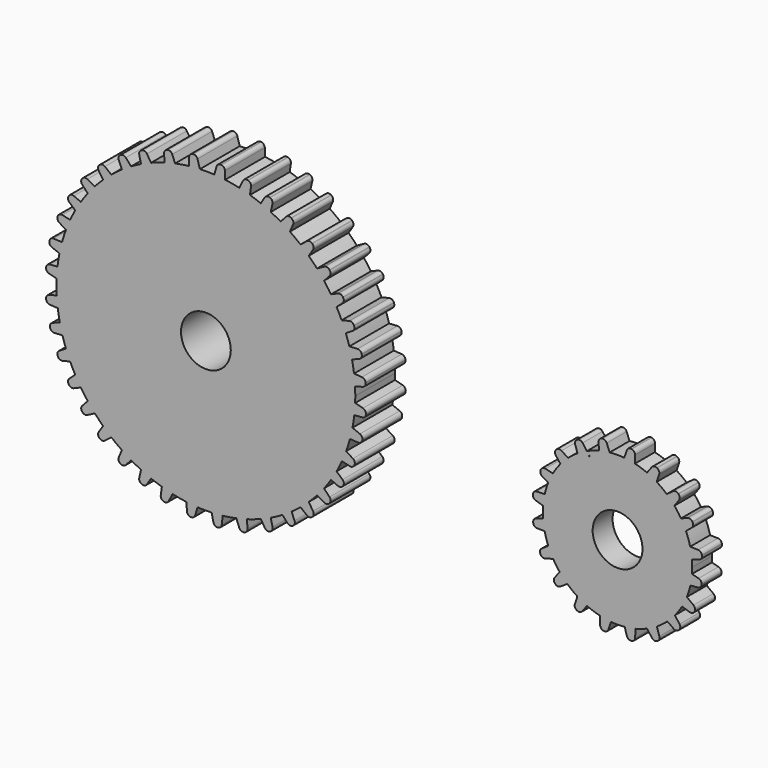
from build123d import *

# Parameters (mm, degrees)
F0_R     = 6.35
F1_DEPTH = 6.35
F2_DEPTH = 12.7


# Not quite as in the source:
# - a feature names something its author has since deleted; it is built from what else it names


with BuildPart() as f1:
    # F0 (on Front) → F1 (new body)
    with BuildSketch(Plane.XZ):
        with BuildLine():
            ThreePointArc((15.9403731731, 16.8749462695), (15.9167372183, 17.7939656764), (15.8458918485, 18.7105551495))
            ThreePointArc((15.8458918485, 18.7105551495), (15.8202944574, 18.7796305883), (15.8049565574, 18.8516818998))
            Line((15.8049565574, 18.8516818998), (15.5952331153, 20.3709607118))
            ThreePointArc((15.5952331153, 20.3709607118), (15.1310569077, 22.1932056362), (14.4780532671, 23.9566177724))
            ThreePointArc((14.4780532671, 23.9566177724), (14.3147953719, 24.0441141766), (14.1936366943, 24.1842189085))
            Line((14.1936366943, 24.1842189085), (13.1956957211, 25.887018151))
            ThreePointArc((13.1956957211, 25.887018151), (13.1258173875, 26.1420313006), (13.1932437417, 26.3977036979))
            ThreePointArc((13.1932437417, 26.3977036979), (12.4320369116, 27.5116667751), (11.5889925331, 28.5650545248))
            ThreePointArc((11.5889925331, 28.5650545248), (11.5056575047, 28.6109888177), (11.43232398, 28.6716261031))
            Line((11.43232398, 28.6716261031), (10.0352798976, 30.0661220051))
            ThreePointArc((10.0352798976, 30.0661220051), (9.9633008227, 30.1564872429), (9.9135443679, 30.2607520913))
            ThreePointArc((9.9135443679, 30.2607520913), (8.6514977587, 31.2798759321), (7.3022744468, 32.1804154933))
            ThreePointArc((7.3022744468, 32.1804154933), (7.2195304339, 32.1994679145), (7.1411027215, 32.232004976))
            Line((7.1411027215, 32.232004976), (5.387230297, 33.1378093871))
            ThreePointArc((5.387230297, 33.1378093871), (5.3110127576, 33.1861782043), (5.2445338397, 33.2472454565))
            ThreePointArc((5.2445338397, 33.2472454565), (3.7183528432, 33.8351149803), (2.1448369807, 34.2810598662))
            ThreePointArc((2.1448369807, 34.2810598662), (0.966155767, 34.5160559457), (-0.2256506981, 34.6713296098))
            ThreePointArc((-0.2256506981, 34.6713296098), (-2.0637768422, 34.7531004215), (-3.9005732165, 34.6455213037))
            ThreePointArc((-3.9005732165, 34.6455213037), (-5.14488714, 34.4636203994), (-6.3733364321, 34.1947014227))
            ThreePointArc((-6.3733364321, 34.1947014227), (-7.7265614442, 33.7905983309), (-9.0436683457, 33.2809448679))
            ThreePointArc((-9.0436683457, 33.2809448679), (-9.1168313714, 33.2490638107), (-9.1898513561, 33.2168564829))
            ThreePointArc((-9.1898513561, 33.2168564829), (-10.4245272255, 32.6111078404), (-11.6089890572, 31.912247275))
            ThreePointArc((-11.6089890572, 31.912247275), (-12.7507583792, 31.1133876767), (-13.8268423682, 30.228030635))
            ThreePointArc((-13.8268423682, 30.228030635), (-14.7493630119, 29.3456648544), (-15.6065697414, 28.399720706))
            ThreePointArc((-15.6065697414, 28.399720706), (-16.565013023, 27.1560522348), (-17.4106440108, 25.8330885078))
            ThreePointArc((-17.4106440108, 25.8330885078), (-18.0360934072, 24.6532938582), (-18.5717424681, 23.4301084893))
            ThreePointArc((-18.5717424681, 23.4301084893), (-19.6223659228, 19.5046246321), (-19.7594034876, 15.4432881694))
            ThreePointArc((-19.7594034876, 15.4432881694), (-19.6255289904, 14.2666276543), (-19.4140506807, 13.1014112481))
            ThreePointArc((-19.4140506807, 13.1014112481), (-18.9881912537, 11.4951039658), (-18.4150278897, 9.9352760603))
            ThreePointArc((-18.4150278897, 9.9352760603), (-15.5468292211, 5.2796901141), (-11.4056163066, 1.7087799079))
            ThreePointArc((-11.4056163066, 1.7087799079), (-10.4078501575, 1.1298023755), (-9.3748229946, 0.6163755043))
            ThreePointArc((-9.3748229946, 0.6163755043), (-7.6230862518, -0.0757609916), (-5.8082549062, -0.5797666777))
            ThreePointArc((-5.8082549062, -0.5797666777), (-2.9905528112, -0.9726518737), (-0.1462043342, -0.9136127831))
            ThreePointArc((-0.1462043342, -0.9136127831), (0.968169079, -0.7658318232), (2.0710524927, -0.5483105786))
            ThreePointArc((2.0710524927, -0.5483105786), (6.3070111873, 1.0111418038), (10.0173898625, 3.5818086203))
            ThreePointArc((10.0173898625, 3.5818086203), (10.9183143035, 4.4510323083), (11.7562031739, 5.3811704212))
            ThreePointArc((11.7562031739, 5.3811704212), (12.7427238301, 6.6713197609), (13.608097106, 8.0456695771))
            ThreePointArc((13.608097106, 8.0456695771), (14.7382278296, 10.4297786161), (15.5051808748, 12.9542497268))
            ThreePointArc((15.5051808748, 12.9542497268), (15.7425331232, 14.2225768426), (15.8877883472, 15.5047198465))
            ThreePointArc((15.8877883472, 15.5047198465), (15.9272221299, 16.189328735), (15.9403731731, 16.8749462695))
        make_face()
        with Locations((-1.9382218483, 16.8749462695)):
            Circle(F0_R, mode=Mode.SUBTRACT)
        with BuildLine():
            Line((5.211917351, 33.8935937172), (5.5737013823, 34.381331087))
            ThreePointArc((5.5737013823, 34.381331087), (4.0553405896, 34.9575265418), (2.4934211396, 35.4023055101))
            Line((2.4934211396, 35.4023055101), (2.4815042905, 34.7500459731))
            ThreePointArc((2.4815042905, 34.7500459731), (2.3862664615, 34.4630802031), (2.1448369807, 34.2810598662))
            ThreePointArc((2.1448369807, 34.2810598662), (3.7183528432, 33.8351149803), (5.2445338397, 33.2472454565))
            ThreePointArc((5.2445338397, 33.2472454565), (5.112336226, 33.5645714945), (5.211917351, 33.8935937172))
        make_face()
        with BuildLine():
            ThreePointArc((5.5737013823, 34.381331087), (6.8331174589, 33.7854786904), (8.045615558, 33.0991716947))
            Line((8.045615558, 33.0991716947), (8.6751480489, 35.0295041106))
            ThreePointArc((8.6751480489, 35.0295041106), (8.6491536191, 35.7302352616), (8.1754346749, 36.2472364398))
            Line((8.1754346749, 36.2472364398), (8.0625950619, 36.3055135515))
            ThreePointArc((8.0625950619, 36.3055135515), (7.3668006059, 36.3925189032), (6.7803620213, 36.0080847178))
            Line((6.7803620213, 36.0080847178), (5.5737013823, 34.381331087))
        make_face()
        with BuildLine():
            ThreePointArc((10.6093123289, 31.2088880188), (11.6215859591, 30.2553092029), (12.5615955235, 29.2304226338))
            Line((12.5615955235, 29.2304226338), (13.7416131662, 30.8728518407))
            ThreePointArc((13.7416131662, 30.8728518407), (13.9291067067, 31.5485337397), (13.6342560751, 32.1847435803))
            Line((13.6342560751, 32.1847435803), (13.5443715775, 32.2744641304))
            ThreePointArc((13.5443715775, 32.2744641304), (12.907624505, 32.5681527784), (12.2322860283, 32.3794259961))
            Line((12.2322860283, 32.3794259961), (10.6093123289, 31.2088880188))
        make_face()
        with BuildLine():
            ThreePointArc((14.2445715458, 26.9258018533), (14.9228666005, 25.7409598225), (15.5145599652, 24.5105802951))
            Line((15.5145599652, 24.5105802951), (16.9847283005, 25.7278830671))
            ThreePointArc((16.9847283005, 25.7278830671), (17.3373273339, 26.3339967346), (17.213323921, 27.0241583172))
            Line((17.213323921, 27.0241583172), (17.1491095982, 27.1337280244))
            ThreePointArc((17.1491095982, 27.1337280244), (16.6075709282, 27.5791892743), (15.9064509254, 27.5677613232))
            Line((15.9064509254, 27.5677613232), (14.2445715458, 26.9258018533))
        make_face()
        with BuildLine():
            Line((7.8588685125, 32.5265501371), (8.045615558, 33.0991716947))
            ThreePointArc((8.045615558, 33.0991716947), (6.8331174589, 33.7854786904), (5.5737013823, 34.381331087))
            Line((5.5737013823, 34.381331087), (5.211917351, 33.8935937172))
            ThreePointArc((5.211917351, 33.8935937172), (5.112336226, 33.5645714945), (5.2445338397, 33.2472454565))
            ThreePointArc((5.2445338397, 33.2472454565), (6.2907108266, 32.7472122379), (7.3022744468, 32.1804154933))
            ThreePointArc((7.3022744468, 32.1804154933), (7.6436669006, 32.252023636), (7.8588685125, 32.5265501371))
        make_face()
        with BuildLine():
            Line((10.0971471144, 30.8394988942), (10.6093123289, 31.2088880188))
            ThreePointArc((10.6093123289, 31.2088880188), (9.3670410612, 32.207706313), (8.045615558, 33.0991716947))
            Line((8.045615558, 33.0991716947), (7.8588685125, 32.5265501371))
            ThreePointArc((7.8588685125, 32.5265501371), (7.6436669006, 32.252023636), (7.3022744468, 32.1804154933))
            ThreePointArc((7.3022744468, 32.1804154933), (8.6514977587, 31.2798759321), (9.9135443679, 30.2607520913))
            ThreePointArc((9.9135443679, 30.2607520913), (9.9096488354, 30.5804845627), (10.0971471144, 30.8394988942))
        make_face()
        with BuildLine():
            Line((12.2055866327, 28.7349051272), (12.5615955235, 29.2304226338))
            ThreePointArc((12.5615955235, 29.2304226338), (11.6215859591, 30.2553092029), (10.6093123289, 31.2088880188))
            Line((10.6093123289, 31.2088880188), (10.0971471144, 30.8394988942))
            ThreePointArc((10.0971471144, 30.8394988942), (9.9096488354, 30.5804845627), (9.9135443679, 30.2607520913))
            ThreePointArc((9.9135443679, 30.2607520913), (10.7795614335, 29.4408584265), (11.5889925331, 28.5650545248))
            ThreePointArc((11.5889925331, 28.5650545248), (11.9272825405, 28.5410989601), (12.2055866327, 28.7349051272))
        make_face()
        with BuildLine():
            Line((14.9576789615, 24.0494815399), (15.5145599652, 24.5105802951))
            ThreePointArc((15.5145599652, 24.5105802951), (14.9228666005, 25.7409598225), (14.2445715458, 26.9258018533))
            Line((14.2445715458, 26.9258018533), (13.4515208521, 26.6194580782))
            ThreePointArc((13.4515208521, 26.6194580782), (13.3033019404, 26.5308037607), (13.1932437417, 26.3977036979))
            ThreePointArc((13.1932437417, 26.3977036979), (13.882799327, 25.2019774879), (14.4780532671, 23.9566177724))
            ThreePointArc((14.4780532671, 23.9566177724), (14.7297303581, 23.9417728385), (14.9576789615, 24.0494815399))
        make_face()
        with BuildLine():
            Line((16.4576547873, 18.4356354476), (17.032365312, 18.6125661343))
            ThreePointArc((17.032365312, 18.6125661343), (16.855905049, 19.9867454546), (16.5800366567, 21.3444654768))
            Line((16.5800366567, 21.3444654768), (16.0543517211, 21.3572440052))
            ThreePointArc((16.0543517211, 21.3572440052), (15.6631069255, 21.1877709424), (15.5387787208, 20.7799277046))
            Line((15.5387787208, 20.7799277046), (15.5952331153, 20.3709607118))
            ThreePointArc((15.5952331153, 20.3709607118), (15.7400671152, 19.543702396), (15.8458918485, 18.7105551495))
            ThreePointArc((15.8458918485, 18.7105551495), (16.0999546714, 18.4577862566), (16.4576547873, 18.4356354476))
        make_face()
        with BuildLine():
            ThreePointArc((16.5800366567, 21.3444654768), (16.855905049, 19.9867454546), (17.032365312, 18.6125661343))
            Line((17.032365312, 18.6125661343), (18.8852186558, 19.1829865462))
            ThreePointArc((18.8852186558, 19.1829865462), (19.4430260062, 19.6078992622), (19.5927342366, 20.2929447367))
            Line((19.5927342366, 20.2929447367), (19.5753676562, 20.4187517392))
            ThreePointArc((19.5753676562, 20.4187517392), (19.2456654685, 21.037618707), (18.5936016163, 21.2955190542))
            Line((18.5936016163, 21.2955190542), (16.5800366567, 21.3444654768))
        make_face()
        with BuildLine():
            ThreePointArc((-0.2362501941, 35.8487648754), (1.1366990671, 35.6751420495), (2.4934211396, 35.4023055101))
            Line((2.4934211396, 35.4023055101), (2.5295959018, 37.3823031931))
            ThreePointArc((2.5295959018, 37.3823031931), (2.2978471914, 38.0469830887), (1.6897210439, 38.4015101217))
            Line((1.6897210439, 38.4015101217), (1.5646400937, 38.4235045736))
            ThreePointArc((1.5646400937, 38.4235045736), (0.874539491, 38.2991622462), (0.4293442375, 37.7574048812))
            Line((0.4293442375, 37.7574048812), (-0.2362501941, 35.8487648754))
        make_face()
        with BuildLine():
            Line((2.4815042905, 34.7500459731), (2.4934211396, 35.4023055101))
            ThreePointArc((2.4934211396, 35.4023055101), (1.1366990671, 35.6751420495), (-0.2362501941, 35.8487648754))
            Line((-0.2362501941, 35.8487648754), (-0.4375833341, 35.2714275851))
            ThreePointArc((-0.4375833341, 35.2714275851), (-0.4369173155, 34.9341903866), (-0.2256506981, 34.6713296098))
            ThreePointArc((-0.2256506981, 34.6713296098), (0.966155767, 34.5160559457), (2.1448369807, 34.2810598662))
            ThreePointArc((2.1448369807, 34.2810598662), (2.3862664615, 34.4630802031), (2.4815042905, 34.7500459731))
        make_face()
        with BuildLine():
            Line((13.4515208521, 26.6194580782), (14.2445715458, 26.9258018533))
            ThreePointArc((14.2445715458, 26.9258018533), (13.4462986215, 28.1096705614), (12.5615955235, 29.2304226338))
            Line((12.5615955235, 29.2304226338), (12.2055866327, 28.7349051272))
            ThreePointArc((12.2055866327, 28.7349051272), (11.9272825405, 28.5410989601), (11.5889925331, 28.5650545248))
            ThreePointArc((11.5889925331, 28.5650545248), (12.4320369116, 27.5116667751), (13.1932437417, 26.3977036979))
            ThreePointArc((13.1932437417, 26.3977036979), (13.3033019404, 26.5308037607), (13.4515208521, 26.6194580782))
        make_face()
        with BuildLine():
            Line((16.0543517211, 21.3572440052), (16.5800366567, 21.3444654768))
            ThreePointArc((16.5800366567, 21.3444654768), (16.1168330162, 22.9509230505), (15.5145599652, 24.5105802951))
            Line((15.5145599652, 24.5105802951), (14.9576789615, 24.0494815399))
            ThreePointArc((14.9576789615, 24.0494815399), (14.7297303581, 23.9417728385), (14.4780532671, 23.9566177724))
            ThreePointArc((14.4780532671, 23.9566177724), (15.1310569077, 22.1932056362), (15.5952331153, 20.3709607118))
            Line((15.5952331153, 20.3709607118), (15.5387787208, 20.7799277046))
            ThreePointArc((15.5387787208, 20.7799277046), (15.6631069255, 21.1877709424), (16.0543517211, 21.3572440052))
        make_face()
        with BuildLine():
            ThreePointArc((17.0520692402, 15.3678482719), (17.0968450709, 16.1208061087), (17.1117781517, 16.8749462695))
            ThreePointArc((17.1117781517, 16.8749462695), (17.0919145859, 17.7446630616), (17.032365312, 18.6125661343))
            Line((17.032365312, 18.6125661343), (16.4576547873, 18.4356354476))
            ThreePointArc((16.4576547873, 18.4356354476), (16.0999546714, 18.4577862566), (15.8458918485, 18.7105551495))
            ThreePointArc((15.8458918485, 18.7105551495), (15.9167372183, 17.7939656764), (15.9403731731, 16.8749462695))
            ThreePointArc((15.9403731731, 16.8749462695), (15.9272221299, 16.189328735), (15.8877883472, 15.5047198465))
            ThreePointArc((15.8877883472, 15.5047198465), (16.080221579, 15.5765788646), (16.2853796102, 15.5663588142))
            Line((16.2853796102, 15.5663588142), (17.0520692402, 15.3678482719))
        make_face()
        with BuildLine():
            ThreePointArc((16.6426361925, 12.6732544115), (16.8956046546, 14.0132196475), (17.0520692402, 15.3678482719))
            Line((17.0520692402, 15.3678482719), (16.2853796102, 15.5663588142))
            ThreePointArc((16.2853796102, 15.5663588142), (16.080221579, 15.5765788646), (15.8877883472, 15.5047198465))
            ThreePointArc((15.8877883472, 15.5047198465), (15.7425331232, 14.2225768426), (15.5051808748, 12.9542497268))
            ThreePointArc((15.5051808748, 12.9542497268), (15.706442946, 12.7078541437), (16.0147860165, 12.62948479))
            Line((16.0147860165, 12.62948479), (16.6426361925, 12.6732544115))
        make_face()
        with BuildLine():
            Line((18.7442948356, 14.9296988467), (17.0520692402, 15.3678482719))
            ThreePointArc((17.0520692402, 15.3678482719), (16.8956046546, 14.0132196475), (16.6426361925, 12.6732544115))
            Line((16.6426361925, 12.6732544115), (18.548636262, 12.8061283115))
            ThreePointArc((18.548636262, 12.8061283115), (19.1883530608, 13.0932907632), (19.4896936277, 13.726452448))
            Line((19.4896936277, 13.726452448), (19.5013456229, 13.8529167948))
            ThreePointArc((19.5013456229, 13.8529167948), (19.320770842, 14.5304805223), (18.7442948356, 14.9296988467))
        make_face()
        with BuildLine():
            ThreePointArc((10.7760157382, 2.688661957), (11.7730874807, 3.6498755141), (12.6976895184, 4.6809888123))
            Line((12.6976895184, 4.6809888123), (12.3266407828, 5.1950005902))
            ThreePointArc((12.3266407828, 5.1950005902), (12.0717577478, 5.3810364618), (11.7562031739, 5.3811704212))
            ThreePointArc((11.7562031739, 5.3811704212), (10.9183143035, 4.4510323083), (10.0173898625, 3.5818086203))
            ThreePointArc((10.0173898625, 3.5818086203), (10.0494398828, 3.3044447024), (10.2229314813, 3.0856785899))
            Line((10.2229314813, 3.0856785899), (10.7760157382, 2.688661957))
        make_face()
        with BuildLine():
            Line((13.8674632274, 3.0605077101), (12.6976895184, 4.6809888123))
            ThreePointArc((12.6976895184, 4.6809888123), (11.7730874807, 3.6498755141), (10.7760157382, 2.688661957))
            Line((10.7760157382, 2.688661957), (12.3615222168, 1.5505488472))
            ThreePointArc((12.3615222168, 1.5505488472), (13.0372826913, 1.3633387044), (13.6733688156, 1.6584561368))
            Line((13.6733688156, 1.6584561368), (13.7630516601, 1.7483782553))
            ThreePointArc((13.7630516601, 1.7483782553), (14.0564732303, 2.385248445), (13.8674632274, 3.0605077101))
        make_face()
        with BuildLine():
            ThreePointArc((8.0692019678, 0.6652587783), (9.4675667842, 1.6168177581), (10.7760157382, 2.688661957))
            Line((10.7760157382, 2.688661957), (10.2229314813, 3.0856785899))
            ThreePointArc((10.2229314813, 3.0856785899), (10.0494398828, 3.3044447024), (10.0173898625, 3.5818086203))
            ThreePointArc((10.0173898625, 3.5818086203), (6.3070111873, 1.0111418038), (2.0710524927, -0.5483105786))
            ThreePointArc((2.0710524927, -0.5483105786), (2.4696248166, -0.6806321117), (2.6323912726, -1.0677702863))
            Line((2.6323912726, -1.0677702863), (2.6167825616, -1.6224707076))
            ThreePointArc((2.6167825616, -1.6224707076), (4.1178055543, -1.186809794), (5.5780625274, -0.6295665539))
            ThreePointArc((5.5780625274, -0.6295665539), (6.847518323, -0.0281087692), (8.0692019678, 0.6652587783))
        make_face()
        with BuildLine():
            Line((8.7211913953, -1.333933233), (8.0692019678, 0.6652587783))
            ThreePointArc((8.0692019678, 0.6652587783), (6.847518323, -0.0281087692), (5.5780625274, -0.6295665539))
            Line((5.5780625274, -0.6295665539), (6.8264053677, -2.3125138402))
            ThreePointArc((6.8264053677, -2.3125138402), (7.4128439523, -2.6969480255), (8.1086384084, -2.6099426739))
            Line((8.1086384084, -2.6099426739), (8.2214780213, -2.5516655622))
            ThreePointArc((8.2214780213, -2.5516655622), (8.6951969656, -2.034664384), (8.7211913953, -1.333933233))
        make_face()
        with BuildLine():
            ThreePointArc((2.6323912726, -1.0677702863), (2.4696248166, -0.6806321117), (2.0710524927, -0.5483105786))
            ThreePointArc((2.0710524927, -0.5483105786), (0.968169079, -0.7658318232), (-0.1462043342, -0.9136127831))
            ThreePointArc((-0.1462043342, -0.9136127831), (-0.307123587, -1.1573602735), (-0.3076320666, -1.4494348983))
            Line((-0.3076320666, -1.4494348983), (-0.1177133596, -2.0878659914))
            ThreePointArc((-0.1177133596, -2.0878659914), (1.2580164677, -1.9050047588), (2.6167825616, -1.6224707076))
            Line((2.6167825616, -1.6224707076), (2.6323912726, -1.0677702863))
        make_face()
        with BuildLine():
            Line((2.558444955, -3.6956652863), (2.6167825616, -1.6224707076))
            ThreePointArc((2.6167825616, -1.6224707076), (1.2580164677, -1.9050047588), (-0.1177133596, -2.0878659914))
            Line((-0.1177133596, -2.0878659914), (0.4430553901, -3.9729473063))
            ThreePointArc((0.4430553901, -3.9729473063), (0.8626431653, -4.5347710822), (1.5462336641, -4.6909885148))
            Line((1.5462336641, -4.6909885148), (1.6722001619, -4.6748193636))
            ThreePointArc((1.6722001619, -4.6748193636), (2.2961158261, -4.3488806081), (2.558444955, -3.6956652863))
        make_face()
        with BuildLine():
            ThreePointArc((-0.3076320666, -1.4494348983), (-0.307123587, -1.1573602735), (-0.1462043342, -0.9136127831))
            ThreePointArc((-0.1462043342, -0.9136127831), (-2.9905528112, -0.9726518737), (-5.8082549062, -0.5797666777))
            ThreePointArc((-5.8082549062, -0.5797666777), (-6.1858467593, -0.7138003118), (-6.34884087, -1.0798242762))
            Line((-6.34884087, -1.0798242762), (-6.3566540147, -1.6555679486))
            ThreePointArc((-6.3566540147, -1.6555679486), (-4.9891450286, -1.9291588075), (-3.6052849825, -2.1019713017))
            ThreePointArc((-3.6052849825, -2.1019713017), (-1.8611756988, -2.1748979264), (-0.1177133596, -2.0878659914))
            Line((-0.1177133596, -2.0878659914), (-0.3076320666, -1.4494348983))
        make_face()
        with BuildLine():
            ThreePointArc((-9.3657178881, -0.005932361), (-9.2641292549, 0.3067745438), (-9.3748229946, 0.6163755043))
            ThreePointArc((-9.3748229946, 0.6163755043), (-10.4078501575, 1.1298023755), (-11.4056163066, 1.7087799079))
            ThreePointArc((-11.4056163066, 1.7087799079), (-11.7711518429, 1.6578694144), (-12.0062843133, 1.3734035499))
            Line((-12.0062843133, 1.3734035499), (-12.1900419119, 0.8187111759))
            ThreePointArc((-12.1900419119, 0.8187111759), (-10.9888325226, 0.1122213592), (-9.7391898097, -0.504564623))
            Line((-9.7391898097, -0.504564623), (-9.3657178881, -0.005932361))
        make_face()
        with BuildLine():
            Line((-10.943977017, -2.1131079583), (-9.7391898097, -0.504564623))
            ThreePointArc((-9.7391898097, -0.504564623), (-10.9888325226, 0.1122213592), (-12.1900419119, 0.8187111759))
            Line((-12.1900419119, 0.8187111759), (-12.834192613, -1.1257280437))
            ThreePointArc((-12.834192613, -1.1257280437), (-12.8114565423, -1.8265724826), (-12.3401465367, -2.345770648))
            Line((-12.3401465367, -2.345770648), (-12.2275791052, -2.4045717821))
            ThreePointArc((-12.2275791052, -2.4045717821), (-11.5321967051, -2.4948113181), (-10.943977017, -2.1131079583))
        make_face()
        with BuildLine():
            ThreePointArc((-12.0062843133, 1.3734035499), (-11.7711518429, 1.6578694144), (-11.4056163066, 1.7087799079))
            ThreePointArc((-11.4056163066, 1.7087799079), (-15.5468292211, 5.2796901141), (-18.4150278897, 9.9352760603))
            ThreePointArc((-18.4150278897, 9.9352760603), (-18.7414212733, 10.154936904), (-19.126932237, 10.0764205102))
            Line((-19.126932237, 10.0764205102), (-19.6058378095, 9.750492168))
            ThreePointArc((-19.6058378095, 9.750492168), (-19.0338930559, 8.4701544244), (-18.369315486, 7.2353580071))
            ThreePointArc((-18.369315486, 7.2353580071), (-17.5775359896, 5.9977061238), (-16.6927272642, 4.8247566474))
            ThreePointArc((-16.6927272642, 4.8247566474), (-15.7640865252, 3.7696814521), (-14.760180976, 2.7859482879))
            ThreePointArc((-14.760180976, 2.7859482879), (-13.5169664696, 1.747647337), (-12.1900419119, 0.8187111759))
            Line((-12.1900419119, 0.8187111759), (-12.0062843133, 1.3734035499))
        make_face()
        with BuildLine():
            Line((-16.5341745213, 1.6175129205), (-14.760180976, 2.7859482879))
            ThreePointArc((-14.760180976, 2.7859482879), (-15.7640865252, 3.7696814521), (-16.6927272642, 4.8247566474))
            Line((-16.6927272642, 4.8247566474), (-17.9782808215, 3.1867137008))
            ThreePointArc((-17.9782808215, 3.1867137008), (-18.1942481937, 2.5195870632), (-17.9266317271, 1.8714502851))
            Line((-17.9266317271, 1.8714502851), (-17.8406313062, 1.7780001508))
            ThreePointArc((-17.8406313062, 1.7780001508), (-17.216906141, 1.4575835865), (-16.5341745213, 1.6175129205))
        make_face()
        with BuildLine():
            ThreePointArc((-6.34884087, -1.0798242762), (-6.1858467593, -0.7138003118), (-5.8082549062, -0.5797666777))
            ThreePointArc((-5.8082549062, -0.5797666777), (-7.6230862518, -0.0757609916), (-9.3748229946, 0.6163755043))
            ThreePointArc((-9.3748229946, 0.6163755043), (-9.2641292549, 0.3067745438), (-9.3657178881, -0.005932361))
            Line((-9.3657178881, -0.005932361), (-9.7391898097, -0.504564623))
            ThreePointArc((-9.7391898097, -0.504564623), (-8.0749666723, -1.1595446566), (-6.3566540147, -1.6555679486))
            Line((-6.3566540147, -1.6555679486), (-6.34884087, -1.0798242762))
        make_face()
        with BuildLine():
            ThreePointArc((-18.369315486, 7.2353580071), (-19.0338930559, 8.4701544244), (-19.6058378095, 9.750492168))
            Line((-19.6058378095, 9.750492168), (-21.3025969916, 8.5957302709))
            ThreePointArc((-21.3025969916, 8.5957302709), (-21.7105405381, 8.0253953524), (-21.6518769185, 7.3266404339))
            Line((-21.6518769185, 7.3266404339), (-21.5982325624, 7.2115262165))
            ThreePointArc((-21.5982325624, 7.2115262165), (-21.1009053231, 6.7171928538), (-20.4018089284, 6.6627494225))
            Line((-20.4018089284, 6.6627494225), (-18.369315486, 7.2353580071))
        make_face()
        with BuildLine():
            ThreePointArc((-19.8874069281, 12.7743021874), (-19.5999528716, 12.8643793737), (-19.4140506807, 13.1014112481))
            ThreePointArc((-19.4140506807, 13.1014112481), (-19.6255289904, 14.2666276543), (-19.7594034876, 15.4432881694))
            ThreePointArc((-19.7594034876, 15.4432881694), (-20.0203238395, 15.6752063624), (-20.3693059404, 15.6839797071))
            Line((-20.3693059404, 15.6839797071), (-20.9379568425, 15.4919892384))
            ThreePointArc((-20.9379568425, 15.4919892384), (-20.7887107897, 14.1251159711), (-20.5412591493, 12.7725685231))
            Line((-20.5412591493, 12.7725685231), (-19.8874069281, 12.7743021874))
        make_face()
        with BuildLine():
            Line((-22.4273979997, 12.7675674977), (-20.5412591493, 12.7725685231))
            ThreePointArc((-20.5412591493, 12.7725685231), (-20.7887107897, 14.1251159711), (-20.9379568425, 15.4919892384))
            Line((-20.9379568425, 15.4919892384), (-22.7758455446, 14.8714730097))
            ThreePointArc((-22.7758455446, 14.8714730097), (-23.321998124, 14.4316807673), (-23.4531887991, 13.7428492472))
            Line((-23.4531887991, 13.7428492472), (-23.432437809, 13.6175560055))
            ThreePointArc((-23.432437809, 13.6175560055), (-23.086175845, 13.0077998996), (-22.4273979997, 12.7675674977))
        make_face()
        with BuildLine():
            ThreePointArc((-19.126932237, 10.0764205102), (-18.7414212733, 10.154936904), (-18.4150278897, 9.9352760603))
            ThreePointArc((-18.4150278897, 9.9352760603), (-18.9881912537, 11.4951039658), (-19.4140506807, 13.1014112481))
            ThreePointArc((-19.4140506807, 13.1014112481), (-19.5999528716, 12.8643793737), (-19.8874069281, 12.7743021874))
            Line((-19.8874069281, 12.7743021874), (-20.5412591493, 12.7725685231))
            ThreePointArc((-20.5412591493, 12.7725685231), (-20.136389569, 11.2420791837), (-19.6058378095, 9.750492168))
            Line((-19.6058378095, 9.750492168), (-19.126932237, 10.0764205102))
        make_face()
        with BuildLine():
            ThreePointArc((-20.3693059404, 15.6839797071), (-20.0203238395, 15.6752063624), (-19.7594034876, 15.4432881694))
            ThreePointArc((-19.7594034876, 15.4432881694), (-19.6223659228, 19.5046246321), (-18.5717424681, 23.4301084893))
            ThreePointArc((-18.5717424681, 23.4301084893), (-18.7640499383, 23.4276918663), (-18.9435363809, 23.4967760187))
            Line((-18.9435363809, 23.4967760187), (-19.6346326455, 23.9275730778))
            ThreePointArc((-19.6346326455, 23.9275730778), (-20.130694126, 22.5261808623), (-20.5159684179, 21.0903741713))
            ThreePointArc((-20.5159684179, 21.0903741713), (-20.7738578895, 19.7247383535), (-20.9314988607, 18.3439351487))
            ThreePointArc((-20.9314988607, 18.3439351487), (-20.9881730084, 16.9180832155), (-20.9379568425, 15.4919892384))
            Line((-20.9379568425, 15.4919892384), (-20.3693059404, 15.6839797071))
        make_face()
        with BuildLine():
            Line((-22.8238103672, 18.9105846672), (-20.9314988607, 18.3439351487))
            ThreePointArc((-20.9314988607, 18.3439351487), (-20.7738578895, 19.7247383535), (-20.5159684179, 21.0903741713))
            Line((-20.5159684179, 21.0903741713), (-22.5484725417, 21.0253005292))
            ThreePointArc((-22.5484725417, 21.0253005292), (-23.1985307246, 20.7623856852), (-23.5234566671, 20.1409977321))
            Line((-23.5234566671, 20.1409977321), (-23.5398537764, 20.0150607049))
            ThreePointArc((-23.5398537764, 20.0150607049), (-23.3848738183, 19.3311885904), (-22.8238103672, 18.9105846672))
        make_face()
        with BuildLine():
            ThreePointArc((-19.6346326455, 23.9275730778), (-19.0803140295, 25.1846499736), (-18.4368367683, 26.3985068285))
            Line((-18.4368367683, 26.3985068285), (-20.3544127833, 26.856521344))
            ThreePointArc((-20.3544127833, 26.856521344), (-21.0507603334, 26.7740595595), (-21.527843848, 26.260161538))
            Line((-21.527843848, 26.260161538), (-21.5768242011, 26.1429867754))
            ThreePointArc((-21.5768242011, 26.1429867754), (-21.6073920144, 25.4424402279), (-21.1768836013, 24.8889401262))
            Line((-21.1768836013, 24.8889401262), (-19.6346326455, 23.9275730778))
        make_face()
        with BuildLine():
            ThreePointArc((-18.9435363809, 23.4967760187), (-18.7640499383, 23.4276918663), (-18.5717424681, 23.4301084893))
            ThreePointArc((-18.5717424681, 23.4301084893), (-18.0360934072, 24.6532938582), (-17.4106440108, 25.8330885078))
            ThreePointArc((-17.4106440108, 25.8330885078), (-17.5405059835, 26.0970492776), (-17.7946936797, 26.2451304548))
            Line((-17.7946936797, 26.2451304548), (-18.4368367683, 26.3985068285))
            ThreePointArc((-18.4368367683, 26.3985068285), (-19.0803140295, 25.1846499736), (-19.6346326455, 23.9275730778))
            Line((-19.6346326455, 23.9275730778), (-18.9435363809, 23.4967760187))
        make_face()
        with BuildLine():
            Line((-16.0585190798, 28.5924233141), (-16.5004518633, 29.1568010557))
            ThreePointArc((-16.5004518633, 29.1568010557), (-17.5297602195, 27.8205586882), (-18.4368367683, 26.3985068285))
            Line((-18.4368367683, 26.3985068285), (-17.7946936797, 26.2451304548))
            ThreePointArc((-17.7946936797, 26.2451304548), (-17.5405059835, 26.0970492776), (-17.4106440108, 25.8330885078))
            ThreePointArc((-17.4106440108, 25.8330885078), (-16.565013023, 27.1560522348), (-15.6065697414, 28.399720706))
            ThreePointArc((-15.6065697414, 28.399720706), (-15.8573235594, 28.4379569694), (-16.0585190798, 28.5924233141))
        make_face()
        with BuildLine():
            Line((-14.0387921961, 30.7822944157), (-14.5710975852, 31.1337313024))
            ThreePointArc((-14.5710975852, 31.1337313024), (-15.5716552939, 30.180283262), (-16.5004518633, 29.1568010557))
            Line((-16.5004518633, 29.1568010557), (-16.0585190798, 28.5924233141))
            ThreePointArc((-16.0585190798, 28.5924233141), (-15.8573235594, 28.4379569694), (-15.6065697414, 28.399720706))
            ThreePointArc((-15.6065697414, 28.399720706), (-14.7493630119, 29.3456648544), (-13.8268423682, 30.228030635))
            ThreePointArc((-13.8268423682, 30.228030635), (-13.8437339218, 30.5392278991), (-14.0387921961, 30.7822944157))
        make_face()
        with BuildLine():
            ThreePointArc((-16.5004518633, 29.1568010557), (-15.5716552939, 30.180283262), (-14.5710975852, 31.1337313024))
            Line((-14.5710975852, 31.1337313024), (-16.2357043874, 32.2327324477))
            ThreePointArc((-16.2357043874, 32.2327324477), (-16.918260633, 32.3934086062), (-17.5423359661, 32.0736745997))
            Line((-17.5423359661, 32.0736745997), (-17.6284385717, 31.9803186073))
            ThreePointArc((-17.6284385717, 31.9803186073), (-17.8967639508, 31.332474994), (-17.681526556, 30.6651124836))
            Line((-17.681526556, 30.6651124836), (-16.5004518633, 29.1568010557))
        make_face()
        with BuildLine():
            Line((-11.9301195305, 32.2367820713), (-12.1623391128, 32.9488358474))
            ThreePointArc((-12.1623391128, 32.9488358474), (-13.4026966899, 32.0890291077), (-14.5710975852, 31.1337313024))
            Line((-14.5710975852, 31.1337313024), (-14.0387921961, 30.7822944157))
            ThreePointArc((-14.0387921961, 30.7822944157), (-13.8437339218, 30.5392278991), (-13.8268423682, 30.228030635))
            ThreePointArc((-13.8268423682, 30.228030635), (-12.7507583792, 31.1133876767), (-11.6089890572, 31.912247275))
            ThreePointArc((-11.6089890572, 31.912247275), (-11.8079655966, 32.0365062994), (-11.9301195305, 32.2367820713))
        make_face()
        with BuildLine():
            ThreePointArc((-12.1623391128, 32.9488358474), (-10.9839985184, 33.6402802785), (-9.7591311474, 34.24549254))
            Line((-9.7591311474, 34.24549254), (-10.8516130394, 35.718316652))
            ThreePointArc((-10.8516130394, 35.718316652), (-11.4380516239, 36.1027508374), (-12.13384608, 36.0157454857))
            Line((-12.13384608, 36.0157454857), (-12.246685693, 35.957468374))
            ThreePointArc((-12.246685693, 35.957468374), (-12.7204046372, 35.4404671958), (-12.7463990669, 34.7397360448))
            Line((-12.7463990669, 34.7397360448), (-12.1623391128, 32.9488358474))
        make_face()
        with BuildLine():
            Line((-9.2831683691, 33.6038256514), (-9.7591311474, 34.24549254))
            ThreePointArc((-9.7591311474, 34.24549254), (-10.9839985184, 33.6402802785), (-12.1623391128, 32.9488358474))
            Line((-12.1623391128, 32.9488358474), (-11.9301195305, 32.2367820713))
            ThreePointArc((-11.9301195305, 32.2367820713), (-11.8079655966, 32.0365062994), (-11.6089890572, 31.912247275))
            ThreePointArc((-11.6089890572, 31.912247275), (-10.4245272255, 32.6111078404), (-9.1898513561, 33.2168564829))
            ThreePointArc((-9.1898513561, 33.2168564829), (-9.1971298424, 33.4198374977), (-9.2831683691, 33.6038256514))
        make_face()
        with BuildLine():
            Line((-6.6266204512, 34.6047185562), (-6.6694460804, 35.3280765532))
            ThreePointArc((-6.6694460804, 35.3280765532), (-8.2375877754, 34.8532801444), (-9.7591311474, 34.24549254))
            Line((-9.7591311474, 34.24549254), (-9.2831683691, 33.6038256514))
            Line((-9.2831683691, 33.6038256514), (-9.0436683457, 33.2809448679))
            ThreePointArc((-9.0436683457, 33.2809448679), (-7.7265614442, 33.7905983309), (-6.3733364321, 34.1947014227))
            ThreePointArc((-6.3733364321, 34.1947014227), (-6.5516958206, 34.3677620914), (-6.6266204512, 34.6047185562))
        make_face()
        with BuildLine():
            Line((-3.7310490512, 35.2411707369), (-3.9588371444, 35.8174807838))
            ThreePointArc((-3.9588371444, 35.8174807838), (-5.3229985587, 35.6218336544), (-6.6694460804, 35.3280765532))
            Line((-6.6694460804, 35.3280765532), (-6.6266204512, 34.6047185562))
            ThreePointArc((-6.6266204512, 34.6047185562), (-6.5516958206, 34.3677620914), (-6.3733364321, 34.1947014227))
            ThreePointArc((-6.3733364321, 34.1947014227), (-5.14488714, 34.4636203994), (-3.9005732165, 34.6455213037))
            ThreePointArc((-3.9005732165, 34.6455213037), (-3.7148491755, 34.9146118509), (-3.7310490512, 35.2411707369))
        make_face()
        with BuildLine():
            ThreePointArc((-6.6694460804, 35.3280765532), (-5.3229985587, 35.6218336544), (-3.9588371444, 35.8174807838))
            Line((-3.9588371444, 35.8174807838), (-4.6988185137, 37.6896536955))
            ThreePointArc((-4.6988185137, 37.6896536955), (-5.1657757993, 38.2127700781), (-5.8603802762, 38.3088142186))
            Line((-5.8603802762, 38.3088142186), (-5.984458199, 38.2817278922))
            ThreePointArc((-5.984458199, 38.2817278922), (-6.5775922415, 37.9026515989), (-6.7819916623, 37.2290584686))
            Line((-6.7819916623, 37.2290584686), (-6.6694460804, 35.3280765532))
        make_face()
        with BuildLine():
            Line((-0.4375833341, 35.2714275851), (-0.2362501941, 35.8487648754))
            ThreePointArc((-0.2362501941, 35.8487648754), (-2.0983096874, 35.9242736037), (-3.9588371444, 35.8174807838))
            Line((-3.9588371444, 35.8174807838), (-3.7310490512, 35.2411707369))
            ThreePointArc((-3.7310490512, 35.2411707369), (-3.7148491755, 34.9146118509), (-3.9005732165, 34.6455213037))
            ThreePointArc((-3.9005732165, 34.6455213037), (-2.0637768422, 34.7531004215), (-0.2256506981, 34.6713296098))
            ThreePointArc((-0.2256506981, 34.6713296098), (-0.4369173155, 34.9341903866), (-0.4375833341, 35.2714275851))
        make_face()
        with BuildLine():
            Line((17.4285609011, 8.4952288689), (15.7362705164, 9.7675684373))
            ThreePointArc((15.7362705164, 9.7675684373), (15.1657140343, 8.4869860094), (14.5025251751, 7.2518315288))
            Line((14.5025251751, 7.2518315288), (16.4377338304, 6.6068179467))
            ThreePointArc((16.4377338304, 6.6068179467), (17.1386185859, 6.6282752513), (17.6586758174, 7.0986371675))
            Line((17.6586758174, 7.0986371675), (17.717682239, 7.2110971258))
            ThreePointArc((17.717682239, 7.2110971258), (17.8091903873, 7.9063137217), (17.4285609011, 8.4952288689))
        make_face()
        with BuildLine():
            ThreePointArc((15.8049565574, 18.8516818998), (15.8202944574, 18.7796305883), (15.8458918485, 18.7105551495))
            ThreePointArc((15.8458918485, 18.7105551495), (15.7400671152, 19.543702396), (15.5952331153, 20.3709607118))
            Line((15.5952331153, 20.3709607118), (15.8049565574, 18.8516818998))
        make_face()
        with BuildLine():
            ThreePointArc((14.1936366943, 24.1842189085), (14.3147953719, 24.0441141766), (14.4780532671, 23.9566177724))
            ThreePointArc((14.4780532671, 23.9566177724), (13.882799327, 25.2019774879), (13.1932437417, 26.3977036979))
            ThreePointArc((13.1932437417, 26.3977036979), (13.1258173875, 26.1420313006), (13.1956957211, 25.887018151))
            Line((13.1956957211, 25.887018151), (14.1936366943, 24.1842189085))
        make_face()
        with BuildLine():
            ThreePointArc((11.43232398, 28.6716261031), (11.5056575047, 28.6109888177), (11.5889925331, 28.5650545248))
            ThreePointArc((11.5889925331, 28.5650545248), (10.7795614335, 29.4408584265), (9.9135443679, 30.2607520913))
            ThreePointArc((9.9135443679, 30.2607520913), (9.9633008227, 30.1564872429), (10.0352798976, 30.0661220051))
            Line((10.0352798976, 30.0661220051), (11.43232398, 28.6716261031))
        make_face()
        with BuildLine():
            ThreePointArc((7.1411027215, 32.232004976), (7.2195304339, 32.1994679145), (7.3022744468, 32.1804154933))
            ThreePointArc((7.3022744468, 32.1804154933), (6.2907108266, 32.7472122379), (5.2445338397, 33.2472454565))
            ThreePointArc((5.2445338397, 33.2472454565), (5.3110127576, 33.1861782043), (5.387230297, 33.1378093871))
            Line((5.387230297, 33.1378093871), (7.1411027215, 32.232004976))
        make_face()
        with BuildLine():
            ThreePointArc((15.7362705164, 9.7675684373), (16.2475792339, 11.2022803178), (16.6426361925, 12.6732544115))
            Line((16.6426361925, 12.6732544115), (16.0147860165, 12.62948479))
            ThreePointArc((16.0147860165, 12.62948479), (15.706442946, 12.7078541437), (15.5051808748, 12.9542497268))
            ThreePointArc((15.5051808748, 12.9542497268), (14.7382278296, 10.4297786161), (13.608097106, 8.0456695771))
            ThreePointArc((13.608097106, 8.0456695771), (13.6556609814, 7.677067901), (13.9410414578, 7.4389765287))
            Line((13.9410414578, 7.4389765287), (14.5025251751, 7.2518315288))
            ThreePointArc((14.5025251751, 7.2518315288), (15.1657140343, 8.4869860094), (15.7362705164, 9.7675684373))
        make_face()
        with BuildLine():
            ThreePointArc((12.6976895184, 4.6809888123), (13.6531854724, 5.9291471776), (14.5025251751, 7.2518315288))
            Line((14.5025251751, 7.2518315288), (13.9410414578, 7.4389765287))
            ThreePointArc((13.9410414578, 7.4389765287), (13.6556609814, 7.677067901), (13.608097106, 8.0456695771))
            ThreePointArc((13.608097106, 8.0456695771), (12.7427238301, 6.6713197609), (11.7562031739, 5.3811704212))
            ThreePointArc((11.7562031739, 5.3811704212), (12.0717577478, 5.3810364618), (12.3266407828, 5.1950005902))
            Line((12.3266407828, 5.1950005902), (12.6976895184, 4.6809888123))
        make_face()
        with BuildLine():
            Line((-4.2825227739, -4.0737472292), (-3.6052849825, -2.1019713017))
            ThreePointArc((-3.6052849825, -2.1019713017), (-4.9891450286, -1.9291588075), (-6.3566540147, -1.6555679486))
            Line((-6.3566540147, -1.6555679486), (-6.3845136197, -3.7085174199))
            ThreePointArc((-6.3845136197, -3.7085174199), (-6.1496445617, -4.3721011403), (-5.5398594306, -4.7237670646))
            Line((-5.5398594306, -4.7237670646), (-5.4146765232, -4.7451735985))
            ThreePointArc((-5.4146765232, -4.7451735985), (-4.7251677424, -4.6175903023), (-4.2825227739, -4.0737472292))
        make_face()
    extrude(amount=F1_DEPTH)


with BuildPart() as f2:
    # F0 (on Front) → F2 (new body)
    with BuildSketch(Plane.XZ):
        with BuildLine():
            Line((-61.7964714273, 29.5273752882), (-63.7883592613, 30.0480118433))
            ThreePointArc((-63.7883592613, 30.0480118433), (-63.8712296553, 28.6564887216), (-64.0049485897, 27.2689285078))
            Line((-64.0049485897, 27.2689285078), (-61.9970211528, 27.4042610891))
            ThreePointArc((-61.9970211528, 27.4042610891), (-61.356644569, 27.6899491833), (-61.0538463059, 28.3224150466))
            Line((-61.0538463059, 28.3224150466), (-61.0419030294, 28.4488522173))
            ThreePointArc((-61.0419030294, 28.4488522173), (-61.2209165548, 29.1268301035), (-61.7964714273, 29.5273752882))
        make_face()
        with BuildLine():
            ThreePointArc((-64.0049485897, 27.2689285078), (-63.8712296553, 28.6564887216), (-63.7883592613, 30.0480118433))
            Line((-63.7883592613, 30.0480118433), (-64.3435971547, 30.1931390634))
            ThreePointArc((-64.3435971547, 30.1931390634), (-64.7642692558, 30.1177147331), (-64.9793090813, 29.7483751608))
            ThreePointArc((-64.9793090813, 29.7483751608), (-65.0493111941, 28.6759002836), (-65.1504971322, 27.6059170763))
            ThreePointArc((-65.1504971322, 27.6059170763), (-64.9552409122, 27.3218285358), (-64.62375825, 27.2272212692))
            Line((-64.62375825, 27.2272212692), (-64.0049485897, 27.2689285078))
        make_face()
        with BuildLine():
            ThreePointArc((-63.7883592613, 30.0480118433), (-63.7641247407, 30.8322672517), (-63.7560454249, 31.6168554127))
            ThreePointArc((-63.7560454249, 31.6168554127), (-63.7715390866, 32.7033069603), (-63.8180074704, 33.78887488))
            Line((-63.8180074704, 33.78887488), (-64.3999147876, 33.6367768472))
            ThreePointArc((-64.3999147876, 33.6367768472), (-64.7635619123, 33.6776336874), (-65.0059051145, 33.9518202753))
            ThreePointArc((-65.0059051145, 33.9518202753), (-64.9504832262, 32.7849224503), (-64.9320030973, 31.6168554127))
            ThreePointArc((-64.9320030973, 31.6168554127), (-64.9438314879, 30.6823159128), (-64.9793090813, 29.7483751608))
            ThreePointArc((-64.9793090813, 29.7483751608), (-64.7642692558, 30.1177147331), (-64.3435971547, 30.1931390634))
            Line((-64.3435971547, 30.1931390634), (-63.7883592613, 30.0480118433))
        make_face()
        with BuildLine():
            ThreePointArc((-64.9320030973, 31.6168554127), (-64.9504832262, 32.7849224503), (-65.0059051145, 33.9518202753))
            ThreePointArc((-65.0059051145, 33.9518202753), (-65.0937911823, 35.0696173237), (-65.2155761828, 36.1842305375))
            ThreePointArc((-65.2155761828, 36.1842305375), (-65.4724798258, 37.9113812968), (-65.8107510139, 39.6244550927))
            ThreePointArc((-65.8107510139, 39.6244550927), (-66.4847950709, 42.2121161552), (-67.3443450265, 44.7442099604))
            ThreePointArc((-67.3443450265, 44.7442099604), (-67.761717545, 45.7929517803), (-68.2109506135, 46.8284462874))
            ThreePointArc((-68.2109506135, 46.8284462874), (-68.8905264984, 48.2499388224), (-69.6301263189, 49.6411456783))
            ThreePointArc((-69.6301263189, 49.6411456783), (-70.2433073558, 50.6961555463), (-70.8910146153, 51.7303277328))
            ThreePointArc((-70.8910146153, 51.7303277328), (-73.558532541, 55.3367977903), (-76.6436951279, 58.5931838195))
            ThreePointArc((-76.6436951279, 58.5931838195), (-78.8904265008, 60.5299190561), (-81.2853688668, 62.280060851))
            ThreePointArc((-81.2853688668, 62.280060851), (-82.2069448381, 62.8786171663), (-83.1459243337, 63.4494844365))
            ThreePointArc((-83.1459243337, 63.4494844365), (-84.5469579842, 64.2325018693), (-85.9806958327, 64.9538945304))
            ThreePointArc((-85.9806958327, 64.9538945304), (-87.0778416092, 65.4545502779), (-88.1907519715, 65.9191098086))
            ThreePointArc((-88.1907519715, 65.9191098086), (-98.7436011986, 68.4094850109), (-109.5648362982, 67.7272340466))
            ThreePointArc((-109.5648362982, 67.7272340466), (-110.7494113026, 67.4538885653), (-111.9243457258, 67.1416950445))
            ThreePointArc((-111.9243457258, 67.1416950445), (-113.7385765858, 66.576694586), (-115.5213388784, 65.9191098086))
            ThreePointArc((-115.5213388784, 65.9191098086), (-116.6342492407, 65.4545502779), (-117.7313950171, 64.9538945304))
            ThreePointArc((-117.7313950171, 64.9538945304), (-119.1651328657, 64.2325018693), (-120.5661665162, 63.4494844365))
            ThreePointArc((-120.5661665162, 63.4494844365), (-121.5051460118, 62.8786171663), (-122.4267219831, 62.280060851))
            ThreePointArc((-122.4267219831, 62.280060851), (-124.821664349, 60.5299190561), (-127.068395722, 58.5931838195))
            ThreePointArc((-127.068395722, 58.5931838195), (-130.1535583089, 55.3367977903), (-132.8210762345, 51.7303277328))
            ThreePointArc((-132.8210762345, 51.7303277328), (-133.468783494, 50.6961555463), (-134.081964531, 49.6411456783))
            ThreePointArc((-134.081964531, 49.6411456783), (-134.8215643515, 48.2499388224), (-135.5011402364, 46.8284462874))
            ThreePointArc((-135.5011402364, 46.8284462874), (-135.9503733049, 45.7929517803), (-136.3677458234, 44.7442099604))
            ThreePointArc((-136.3677458234, 44.7442099604), (-137.7408713629, 40.3153707582), (-138.5481060805, 35.7493590919))
            ThreePointArc((-138.5481060805, 35.7493590919), (-138.6656316787, 34.5218961421), (-138.7421063969, 33.2911934254))
            ThreePointArc((-138.7421063969, 33.2911934254), (-138.7786059033, 31.2860540642), (-138.7061857354, 29.2818905502))
            ThreePointArc((-138.7061857354, 29.2818905502), (-138.6182996675, 28.1640935017), (-138.496514667, 27.049480288))
            ThreePointArc((-138.496514667, 27.049480288), (-138.2396110241, 25.3223295287), (-137.9013398359, 23.6092557327))
            ThreePointArc((-137.9013398359, 23.6092557327), (-137.227295779, 21.0215946703), (-136.3677458234, 18.489500865))
            ThreePointArc((-136.3677458234, 18.489500865), (-135.9503733049, 17.4407590451), (-135.5011402364, 16.405264538))
            ThreePointArc((-135.5011402364, 16.405264538), (-134.8215643515, 14.983772003), (-134.081964531, 13.5925651471))
            ThreePointArc((-134.081964531, 13.5925651471), (-133.468783494, 12.5375552792), (-132.8210762345, 11.5033830926))
            ThreePointArc((-132.8210762345, 11.5033830926), (-130.1535583089, 7.8969130352), (-127.068395722, 4.6405270059))
            ThreePointArc((-127.068395722, 4.6405270059), (-124.821664349, 2.7037917694), (-122.4267219831, 0.9536499744))
            ThreePointArc((-122.4267219831, 0.9536499744), (-121.5051460118, 0.3550936591), (-120.5661665162, -0.215773611))
            ThreePointArc((-120.5661665162, -0.215773611), (-119.1651328657, -0.9987910438), (-117.7313950171, -1.720183705))
            ThreePointArc((-117.7313950171, -1.720183705), (-116.6342492407, -2.2208394525), (-115.5213388784, -2.6853989832))
            ThreePointArc((-115.5213388784, -2.6853989832), (-101.8560454249, -5.3071869149), (-88.1907519715, -2.6853989832))
            ThreePointArc((-88.1907519715, -2.6853989832), (-87.0778416092, -2.2208394525), (-85.9806958327, -1.720183705))
            ThreePointArc((-85.9806958327, -1.720183705), (-84.4198120088, -0.9309965298), (-82.8980517546, -0.0687782058))
            ThreePointArc((-82.8980517546, -0.0687782058), (-81.8015276632, 0.6136101123), (-80.7295390604, 1.3339290244))
            ThreePointArc((-80.7295390604, 1.3339290244), (-78.6277048314, 2.9144322557), (-76.6436951279, 4.6405270059))
            ThreePointArc((-76.6436951279, 4.6405270059), (-73.558532541, 7.8969130352), (-70.8910146153, 11.5033830926))
            ThreePointArc((-70.8910146153, 11.5033830926), (-70.2433073558, 12.5375552792), (-69.6301263189, 13.5925651471))
            ThreePointArc((-69.6301263189, 13.5925651471), (-68.8406731625, 15.082947944), (-68.1201011214, 16.6078260051))
            ThreePointArc((-68.1201011214, 16.6078260051), (-67.7021935827, 17.5847740935), (-67.3125702326, 18.573342717))
            ThreePointArc((-67.3125702326, 18.573342717), (-66.3976725769, 21.316918676), (-65.7003089279, 24.1236838434))
            ThreePointArc((-65.7003089279, 24.1236838434), (-65.3838204808, 25.8582349673), (-65.1504971322, 27.6059170763))
            ThreePointArc((-65.1504971322, 27.6059170763), (-65.0493111941, 28.6759002836), (-64.9793090813, 29.7483751608))
            ThreePointArc((-64.9793090813, 29.7483751608), (-64.9438314879, 30.6823159128), (-64.9320030973, 31.6168554127))
        make_face()
        with Locations((-101.8560454249, 31.6168554127)):
            Circle(F0_R, mode=Mode.SUBTRACT)
        with BuildLine():
            Line((-64.3999147876, 33.6367768472), (-63.8180074704, 33.78887488))
            ThreePointArc((-63.8180074704, 33.78887488), (-63.9228270689, 35.1778868862), (-64.0783513319, 36.5621389245))
            Line((-64.0783513319, 36.5621389245), (-64.6800758829, 36.6026946414))
            ThreePointArc((-64.6800758829, 36.6026946414), (-65.0278527388, 36.4958711942), (-65.2155761828, 36.1842305375))
            ThreePointArc((-65.2155761828, 36.1842305375), (-65.0937911823, 35.0696173237), (-65.0059051145, 33.9518202753))
            ThreePointArc((-65.0059051145, 33.9518202753), (-64.7635619123, 33.6776336874), (-64.3999147876, 33.6367768472))
        make_face()
        with BuildLine():
            ThreePointArc((-64.0783513319, 36.5621389245), (-63.9228270689, 35.1778868862), (-63.8180074704, 33.78887488))
            Line((-63.8180074704, 33.78887488), (-61.8527890603, 34.3025406224))
            ThreePointArc((-61.8527890603, 34.3025406224), (-61.2772341877, 34.7030858071), (-61.0982206623, 35.3810636933))
            Line((-61.0982206623, 35.3810636933), (-61.1101639388, 35.507500864))
            ThreePointArc((-61.1101639388, 35.507500864), (-61.4129622019, 36.1399667273), (-62.0533387858, 36.4256548215))
            Line((-62.0533387858, 36.4256548215), (-64.0783513319, 36.5621389245))
        make_face()
        with BuildLine():
            ThreePointArc((-64.4718670908, 24.2661268583), (-64.2084576949, 25.7628706066), (-64.0049485897, 27.2689285078))
            Line((-64.0049485897, 27.2689285078), (-64.62375825, 27.2272212692))
            ThreePointArc((-64.62375825, 27.2272212692), (-64.9552409122, 27.3218285358), (-65.1504971322, 27.6059170763))
            ThreePointArc((-65.1504971322, 27.6059170763), (-65.3838204808, 25.8582349673), (-65.7003089279, 24.1236838434))
            ThreePointArc((-65.7003089279, 24.1236838434), (-65.4401453771, 24.4627542978), (-65.0133032868, 24.4841943589))
            Line((-65.0133032868, 24.4841943589), (-64.4718670908, 24.2661268583))
        make_face()
        with BuildLine():
            ThreePointArc((-65.1115707685, 21.544438512), (-64.7667451429, 22.8994128642), (-64.4718670908, 24.2661268583))
            Line((-64.4718670908, 24.2661268583), (-65.0133032868, 24.4841943589))
            ThreePointArc((-65.0133032868, 24.4841943589), (-65.4401453771, 24.4627542978), (-65.7003089279, 24.1236838434))
            ThreePointArc((-65.7003089279, 24.1236838434), (-66.3976725769, 21.316918676), (-67.3125702326, 18.573342717))
            ThreePointArc((-67.3125702326, 18.573342717), (-66.995411608, 18.8373488716), (-66.5868005932, 18.7796784168))
            Line((-66.5868005932, 18.7796784168), (-66.0950038201, 18.473115331))
            ThreePointArc((-66.0950038201, 18.473115331), (-65.5707766703, 19.9983670687), (-65.1115707685, 21.544438512))
        make_face()
        with BuildLine():
            Line((-62.571234932, 23.50063296), (-64.4718670908, 24.2661268583))
            ThreePointArc((-64.4718670908, 24.2661268583), (-64.7667451429, 22.8994128642), (-65.1115707685, 21.544438512))
            Line((-65.1115707685, 21.544438512), (-63.0395436772, 21.4201231633))
            ThreePointArc((-63.0395436772, 21.4201231633), (-62.3680945498, 21.6222516512), (-61.9874964607, 22.2111870898))
            Line((-61.9874964607, 22.2111870898), (-61.9596074132, 22.3350870536))
            ThreePointArc((-61.9596074132, 22.3350870536), (-62.051152625, 23.03029877), (-62.571234932, 23.50063296))
        make_face()
        with BuildLine():
            Line((-64.6800758829, 36.6026946414), (-64.0783513319, 36.5621389245))
            ThreePointArc((-64.0783513319, 36.5621389245), (-64.3055417498, 38.0643102397), (-64.5924393893, 39.5562297721))
            Line((-64.5924393893, 39.5562297721), (-65.1448120185, 39.3337575408))
            ThreePointArc((-65.1448120185, 39.3337575408), (-65.5387609209, 39.3394127994), (-65.8107510139, 39.6244550927))
            ThreePointArc((-65.8107510139, 39.6244550927), (-65.4724798258, 37.9113812968), (-65.2155761828, 36.1842305375))
            ThreePointArc((-65.2155761828, 36.1842305375), (-65.0278527388, 36.4958711942), (-64.6800758829, 36.6026946414))
        make_face()
        with BuildLine():
            Line((-65.1448120185, 39.3337575408), (-64.5924393893, 39.5562297721))
            ThreePointArc((-64.5924393893, 39.5562297721), (-64.9093475998, 40.9201623418), (-65.2761610702, 42.2715285937))
            ThreePointArc((-65.2761610702, 42.2715285937), (-65.6948154507, 43.615832317), (-66.1628542318, 44.9437493663))
            Line((-66.1628542318, 44.9437493663), (-66.6735742631, 44.6253904072))
            ThreePointArc((-66.6735742631, 44.6253904072), (-67.0317545651, 44.5561162618), (-67.3443450265, 44.7442099604))
            ThreePointArc((-67.3443450265, 44.7442099604), (-66.4847950709, 42.2121161552), (-65.8107510139, 39.6244550927))
            ThreePointArc((-65.8107510139, 39.6244550927), (-65.5387609209, 39.3394127994), (-65.1448120185, 39.3337575408))
        make_face()
        with BuildLine():
            ThreePointArc((-65.2761610702, 42.2715285937), (-64.9093475998, 40.9201623418), (-64.5924393893, 39.5562297721))
            Line((-64.5924393893, 39.5562297721), (-62.7027436636, 40.3173189397))
            ThreePointArc((-62.7027436636, 40.3173189397), (-62.1826613566, 40.7876531297), (-62.0911161448, 41.4828648461))
            Line((-62.0911161448, 41.4828648461), (-62.1190051923, 41.6067648099))
            ThreePointArc((-62.1190051923, 41.6067648099), (-62.4996032814, 42.1957002485), (-63.1710524088, 42.3978287364))
            Line((-63.1710524088, 42.3978287364), (-65.2761610702, 42.2715285937))
        make_face()
        with BuildLine():
            Line((-66.6735742631, 44.6253904072), (-66.1628542318, 44.9437493663))
            ThreePointArc((-66.1628542318, 44.9437493663), (-66.6737195129, 46.2392335853), (-67.2315862423, 47.5151831961))
            Line((-67.2315862423, 47.5151831961), (-67.8225378163, 47.3740339553))
            ThreePointArc((-67.8225378163, 47.3740339553), (-68.1190602738, 47.1740805996), (-68.2109506135, 46.8284462874))
            ThreePointArc((-68.2109506135, 46.8284462874), (-67.761717545, 45.7929517803), (-67.3443450265, 44.7442099604))
            ThreePointArc((-67.3443450265, 44.7442099604), (-67.0317545651, 44.5561162618), (-66.6735742631, 44.6253904072))
        make_face()
        with BuildLine():
            ThreePointArc((-67.2315862423, 47.5151831961), (-66.6737195129, 46.2392335853), (-66.1628542318, 44.9437493663))
            Line((-66.1628542318, 44.9437493663), (-64.4394000584, 46.0180700179))
            ThreePointArc((-64.4394000584, 46.0180700179), (-64.0088916452, 46.5715701197), (-64.0394594585, 47.2721166671))
            Line((-64.0394594585, 47.2721166671), (-64.0884398117, 47.3892914298))
            ThreePointArc((-64.0884398117, 47.3892914298), (-64.5655233263, 47.9031894512), (-65.2618708763, 47.9856512358))
            Line((-65.2618708763, 47.9856512358), (-67.2315862423, 47.5151831961))
        make_face()
        with BuildLine():
            ThreePointArc((-69.9529874889, 52.4448388565), (-69.2165284265, 51.2706573377), (-68.5232648047, 50.0704657945))
            Line((-68.5232648047, 50.0704657945), (-67.0178108119, 51.4230111458))
            ThreePointArc((-67.0178108119, 51.4230111458), (-66.689957073, 52.0428593387), (-66.8417091238, 52.7274549649))
            Line((-66.8417091238, 52.7274549649), (-66.9102925394, 52.8343442306))
            ThreePointArc((-66.9102925394, 52.8343442306), (-67.4693655383, 53.2575903034), (-68.1694533429, 53.2178798251))
            Line((-68.1694533429, 53.2178798251), (-69.9529874889, 52.4448388565))
        make_face()
        with BuildLine():
            Line((-68.9762066138, 49.6635291885), (-68.5232648047, 50.0704657945))
            ThreePointArc((-68.5232648047, 50.0704657945), (-69.2165284265, 51.2706573377), (-69.9529874889, 52.4448388565))
            Line((-69.9529874889, 52.4448388565), (-70.5850117722, 52.1708992376))
            ThreePointArc((-70.5850117722, 52.1708992376), (-70.8007305888, 51.9941744078), (-70.8910146153, 51.7303277328))
            ThreePointArc((-70.8910146153, 51.7303277328), (-70.2433073558, 50.6961555463), (-69.6301263189, 49.6411456783))
            ThreePointArc((-69.6301263189, 49.6411456783), (-69.2990955414, 49.5334080056), (-68.9762066138, 49.6635291885))
        make_face()
        with BuildLine():
            Line((-70.5850117722, 52.1708992376), (-69.9529874889, 52.4448388565))
            ThreePointArc((-69.9529874889, 52.4448388565), (-70.8114612471, 53.7040415898), (-71.7196061841, 54.9279049361))
            ThreePointArc((-71.7196061841, 54.9279049361), (-72.5989578704, 56.0224455065), (-73.5180405216, 57.0838434188))
            ThreePointArc((-73.5180405216, 57.0838434188), (-74.5518364875, 58.189212747), (-75.62871727, 59.2526520875))
            Line((-75.62871727, 59.2526520875), (-75.9547072845, 58.751868615))
            ThreePointArc((-75.9547072845, 58.751868615), (-76.2671709433, 58.5334551631), (-76.6436951279, 58.5931838195))
            ThreePointArc((-76.6436951279, 58.5931838195), (-73.558532541, 55.3367977903), (-70.8910146153, 51.7303277328))
            ThreePointArc((-70.8910146153, 51.7303277328), (-70.8007305888, 51.9941744078), (-70.5850117722, 52.1708992376))
        make_face()
        with BuildLine():
            ThreePointArc((-73.5180405216, 57.0838434188), (-72.5989578704, 56.0224455065), (-71.7196061841, 54.9279049361))
            Line((-71.7196061841, 54.9279049361), (-70.3268911628, 56.4181455407))
            ThreePointArc((-70.3268911628, 56.4181455407), (-70.0543083359, 57.0642093601), (-70.2651493647, 57.7329738306))
            Line((-70.2651493647, 57.7329738306), (-70.3427878129, 57.8334789118))
            ThreePointArc((-70.3427878129, 57.8334789118), (-70.9366216962, 58.2063879831), (-71.6305844591, 58.1058119425))
            Line((-71.6305844591, 58.1058119425), (-73.5180405216, 57.0838434188))
        make_face()
        with BuildLine():
            ThreePointArc((-77.7249648157, 61.1007654084), (-76.6598906781, 60.1959349286), (-75.62871727, 59.2526520875))
            Line((-75.62871727, 59.2526520875), (-74.5184296414, 60.9582678099))
            ThreePointArc((-74.5184296414, 60.9582678099), (-74.3621757651, 61.6418499794), (-74.6859433765, 62.2638422544))
            Line((-74.6859433765, 62.2638422544), (-74.7798548465, 62.3493386626))
            ThreePointArc((-74.7798548465, 62.3493386626), (-75.4294220393, 62.6134642355), (-76.0953771024, 62.3939108018))
            Line((-76.0953771024, 62.3939108018), (-77.7249648157, 61.1007654084))
        make_face()
        with BuildLine():
            ThreePointArc((-81.2853688668, 62.280060851), (-78.8904265008, 60.5299190561), (-76.6436951279, 58.5931838195))
            ThreePointArc((-76.6436951279, 58.5931838195), (-76.2671709433, 58.5334551631), (-75.9547072845, 58.751868615))
            Line((-75.9547072845, 58.751868615), (-75.62871727, 59.2526520875))
            ThreePointArc((-75.62871727, 59.2526520875), (-76.6598906781, 60.1959349286), (-77.7249648157, 61.1007654084))
            ThreePointArc((-77.7249648157, 61.1007654084), (-79.0522305028, 62.1389134199), (-80.4241010227, 63.117359522))
            Line((-80.4241010227, 63.117359522), (-80.6593538244, 62.5648157074))
            ThreePointArc((-80.6593538244, 62.5648157074), (-80.9170250233, 62.3007849715), (-81.2853688668, 62.280060851))
        make_face()
        with BuildLine():
            ThreePointArc((-83.1459243337, 63.4494844365), (-82.2069448381, 62.8786171663), (-81.2853688668, 62.280060851))
            ThreePointArc((-81.2853688668, 62.280060851), (-80.9170250233, 62.3007849715), (-80.6593538244, 62.5648157074))
            Line((-80.6593538244, 62.5648157074), (-80.4241010227, 63.117359522))
            ThreePointArc((-80.4241010227, 63.117359522), (-81.5907606982, 63.8802748679), (-82.7845476161, 64.6000021899))
            Line((-82.7845476161, 64.6000021899), (-83.1770868389, 64.1573542684))
            ThreePointArc((-83.1770868389, 64.1573542684), (-83.3048181229, 63.7971103144), (-83.1459243337, 63.4494844365))
        make_face()
        with BuildLine():
            ThreePointArc((-82.7845476161, 64.6000021899), (-81.5907606982, 63.8802748679), (-80.4241010227, 63.117359522))
            Line((-80.4241010227, 63.117359522), (-79.6280336654, 64.9871017361))
            ThreePointArc((-79.6280336654, 64.9871017361), (-79.5928564346, 65.6874319573), (-80.0197131135, 66.2437531164))
            Line((-80.0197131135, 66.2437531164), (-80.1270441527, 66.3116430863))
            ThreePointArc((-80.1270441527, 66.3116430863), (-80.8126078848, 66.458959839), (-81.4303205404, 66.1271000322))
            Line((-81.4303205404, 66.1271000322), (-82.7845476161, 64.6000021899))
        make_face()
        with BuildLine():
            ThreePointArc((-85.9806958327, 64.9538945304), (-84.5469579842, 64.2325018693), (-83.1459243337, 63.4494844365))
            ThreePointArc((-83.1459243337, 63.4494844365), (-83.3048181229, 63.7971103144), (-83.1770868389, 64.1573542684))
            Line((-83.1770868389, 64.1573542684), (-82.7845476161, 64.6000021899))
            ThreePointArc((-82.7845476161, 64.6000021899), (-84.0369142143, 65.2930868363), (-85.3144305632, 65.9386411729))
            Line((-85.3144305632, 65.9386411729), (-85.4517155392, 65.3469409499))
            ThreePointArc((-85.4517155392, 65.3469409499), (-85.6440468757, 65.0533030312), (-85.9806958327, 64.9538945304))
        make_face()
        with BuildLine():
            ThreePointArc((-87.8555819278, 67.051259907), (-86.5748766957, 66.518085796), (-85.3144305632, 65.9386411729))
            Line((-85.3144305632, 65.9386411729), (-84.8566890055, 67.9115138772))
            ThreePointArc((-84.8566890055, 67.9115138772), (-84.9436572625, 68.6073129708), (-85.4606331848, 69.0810594769))
            Line((-85.4606331848, 69.0810594769), (-85.5781225939, 69.1292802063))
            ThreePointArc((-85.5781225939, 69.1292802063), (-86.2788523581, 69.1553119938), (-86.8295537198, 68.7212292061))
            Line((-86.8295537198, 68.7212292061), (-87.8555819278, 67.051259907))
        make_face()
        with BuildLine():
            ThreePointArc((-88.1907519715, 65.9191098086), (-87.0778416092, 65.4545502779), (-85.9806958327, 64.9538945304))
            ThreePointArc((-85.9806958327, 64.9538945304), (-85.6440468757, 65.0533030312), (-85.4517155392, 65.3469409499))
            Line((-85.4517155392, 65.3469409499), (-85.3144305632, 65.9386411729))
            ThreePointArc((-85.3144305632, 65.9386411729), (-86.5748766957, 66.518085796), (-87.8555819278, 67.051259907))
            Line((-87.8555819278, 67.051259907), (-88.2077399509, 66.478085522))
            ThreePointArc((-88.2077399509, 66.478085522), (-88.2828499462, 66.1960568344), (-88.1907519715, 65.9191098086))
        make_face()
        with BuildLine():
            ThreePointArc((-109.5648362982, 67.7272340466), (-98.7436011986, 68.4094850109), (-88.1907519715, 65.9191098086))
            ThreePointArc((-88.1907519715, 65.9191098086), (-88.2828499462, 66.1960568344), (-88.2077399509, 66.478085522))
            Line((-88.2077399509, 66.478085522), (-87.8555819278, 67.051259907))
            ThreePointArc((-87.8555819278, 67.051259907), (-89.2314201425, 67.5644399836), (-90.6260115242, 68.0242219556))
            ThreePointArc((-90.6260115242, 68.0242219556), (-91.9757820837, 68.4134639019), (-93.338984358, 68.7526827333))
            ThreePointArc((-93.338984358, 68.7526827333), (-95.1256746252, 69.1176835222), (-96.9277834726, 69.3967738103))
            ThreePointArc((-96.9277834726, 69.3967738103), (-98.3222707563, 69.5526226594), (-99.7215510568, 69.6570175285))
            ThreePointArc((-99.7215510568, 69.6570175285), (-101.5517104032, 69.7156399103), (-103.3825727009, 69.6862619549))
            ThreePointArc((-103.3825727009, 69.6862619549), (-104.7885100795, 69.6038354328), (-106.1904405907, 69.469504178))
            ThreePointArc((-106.1904405907, 69.469504178), (-107.962749899, 69.2242770269), (-109.7215921714, 68.8961147184))
            Line((-109.7215921714, 68.8961147184), (-109.468683056, 68.2562478047))
            ThreePointArc((-109.468683056, 68.2562478047), (-109.4412428573, 67.9780150311), (-109.5648362982, 67.7272340466))
        make_face()
        with BuildLine():
            ThreePointArc((-93.338984358, 68.7526827333), (-91.9757820837, 68.4134639019), (-90.6260115242, 68.0242219556))
            Line((-90.6260115242, 68.0242219556), (-90.3398676777, 70.0442456949))
            ThreePointArc((-90.3398676777, 70.0442456949), (-90.4871478811, 70.7298172798), (-91.0434462826, 71.156703617))
            Line((-91.0434462826, 71.156703617), (-91.1646913225, 71.1945009753))
            ThreePointArc((-91.1646913225, 71.1945009753), (-91.8650234181, 71.1593610809), (-92.3757963871, 70.6789333231))
            Line((-92.3757963871, 70.6789333231), (-93.338984358, 68.7526827333))
        make_face()
        with BuildLine():
            ThreePointArc((-99.7215510568, 69.6570175285), (-98.3222707563, 69.5526226594), (-96.9277834726, 69.3967738103))
            Line((-96.9277834726, 69.3967738103), (-96.9967260933, 71.4347879375))
            ThreePointArc((-96.9967260933, 71.4347879375), (-97.2608170359, 72.0843692106), (-97.8827920491, 72.4081699815))
            Line((-97.8827920491, 72.4081699815), (-98.0087585469, 72.4243391327))
            ThreePointArc((-98.0087585469, 72.4243391327), (-98.6923490457, 72.2681217001), (-99.1119368209, 71.7062979242))
            Line((-99.1119368209, 71.7062979242), (-99.7215510568, 69.6570175285))
        make_face()
        with BuildLine():
            Line((-106.1213790951, 71.5110323688), (-106.1904405907, 69.469504178))
            ThreePointArc((-106.1904405907, 69.469504178), (-104.7885100795, 69.6038354328), (-103.3825727009, 69.6862619549))
            Line((-103.3825727009, 69.6862619549), (-104.0061683675, 71.7825423555))
            ThreePointArc((-104.0061683675, 71.7825423555), (-104.4257561428, 72.3443661314), (-105.1093466416, 72.500583564))
            Line((-105.1093466416, 72.500583564), (-105.2353131393, 72.4844144128))
            ThreePointArc((-105.2353131393, 72.4844144128), (-105.8572881526, 72.1606136419), (-106.1213790951, 71.5110323688))
        make_face()
        with BuildLine():
            ThreePointArc((-112.411605573, 68.2254630066), (-111.0727009048, 68.5852643826), (-109.7215921714, 68.8961147184))
            Line((-109.7215921714, 68.8961147184), (-110.4364137285, 70.7046326235))
            ThreePointArc((-110.4364137285, 70.7046326235), (-110.9033710141, 71.2277490061), (-111.597975491, 71.3237931466))
            Line((-111.597975491, 71.3237931466), (-111.7220534138, 71.2967068202))
            ThreePointArc((-111.7220534138, 71.2967068202), (-112.3134405277, 70.9199295147), (-112.5199117861, 70.2498030522))
            Line((-112.5199117861, 70.2498030522), (-112.411605573, 68.2254630066))
        make_face()
        with BuildLine():
            ThreePointArc((-117.7313950171, 64.9538945304), (-116.6342492407, 65.4545502779), (-115.5213388784, 65.9191098086))
            ThreePointArc((-115.5213388784, 65.9191098086), (-115.4292409037, 66.1960568344), (-115.5043508989, 66.478085522))
            Line((-115.5043508989, 66.478085522), (-115.8565089221, 67.051259907))
            ThreePointArc((-115.8565089221, 67.051259907), (-117.1372141542, 66.518085796), (-118.3976602866, 65.9386411729))
            Line((-118.3976602866, 65.9386411729), (-118.2603753107, 65.3469409499))
            ThreePointArc((-118.2603753107, 65.3469409499), (-118.0680439742, 65.0533030312), (-117.7313950171, 64.9538945304))
        make_face()
        with BuildLine():
            ThreePointArc((-118.3976602866, 65.9386411729), (-117.1372141542, 66.518085796), (-115.8565089221, 67.051259907))
            Line((-115.8565089221, 67.051259907), (-116.8825371301, 68.7212292061))
            ThreePointArc((-116.8825371301, 68.7212292061), (-117.4332384918, 69.1553119938), (-118.1339682559, 69.1292802063))
            Line((-118.1339682559, 69.1292802063), (-118.2514576651, 69.0810594769))
            ThreePointArc((-118.2514576651, 69.0810594769), (-118.7684335874, 68.6073129708), (-118.8554018444, 67.9115138772))
            Line((-118.8554018444, 67.9115138772), (-118.3976602866, 65.9386411729))
        make_face()
        with BuildLine():
            ThreePointArc((-120.5661665162, 63.4494844365), (-119.1651328657, 64.2325018693), (-117.7313950171, 64.9538945304))
            ThreePointArc((-117.7313950171, 64.9538945304), (-118.0680439742, 65.0533030312), (-118.2603753107, 65.3469409499))
            Line((-118.2603753107, 65.3469409499), (-118.3976602866, 65.9386411729))
            ThreePointArc((-118.3976602866, 65.9386411729), (-119.6751766356, 65.2930868363), (-120.9275432338, 64.6000021899))
            Line((-120.9275432338, 64.6000021899), (-120.5350040109, 64.1573542684))
            ThreePointArc((-120.5350040109, 64.1573542684), (-120.407272727, 63.7971103144), (-120.5661665162, 63.4494844365))
        make_face()
        with BuildLine():
            ThreePointArc((-123.2879898272, 63.117359522), (-122.1213301517, 63.8802748679), (-120.9275432338, 64.6000021899))
            Line((-120.9275432338, 64.6000021899), (-122.2817703094, 66.1271000322))
            ThreePointArc((-122.2817703094, 66.1271000322), (-122.8994829651, 66.458959839), (-123.5850466971, 66.3116430863))
            Line((-123.5850466971, 66.3116430863), (-123.6923777363, 66.2437531164))
            ThreePointArc((-123.6923777363, 66.2437531164), (-124.1192344153, 65.6874319573), (-124.0840571845, 64.9871017361))
            Line((-124.0840571845, 64.9871017361), (-123.2879898272, 63.117359522))
        make_face()
        with BuildLine():
            ThreePointArc((-122.4267219831, 62.280060851), (-121.5051460118, 62.8786171663), (-120.5661665162, 63.4494844365))
            ThreePointArc((-120.5661665162, 63.4494844365), (-120.407272727, 63.7971103144), (-120.5350040109, 64.1573542684))
            Line((-120.5350040109, 64.1573542684), (-120.9275432338, 64.6000021899))
            ThreePointArc((-120.9275432338, 64.6000021899), (-122.1213301517, 63.8802748679), (-123.2879898272, 63.117359522))
            Line((-123.2879898272, 63.117359522), (-123.0527370255, 62.5648157074))
            ThreePointArc((-123.0527370255, 62.5648157074), (-122.7950658266, 62.3007849715), (-122.4267219831, 62.280060851))
        make_face()
        with BuildLine():
            ThreePointArc((-127.068395722, 58.5931838195), (-124.821664349, 60.5299190561), (-122.4267219831, 62.280060851))
            ThreePointArc((-122.4267219831, 62.280060851), (-122.7950658266, 62.3007849715), (-123.0527370255, 62.5648157074))
            Line((-123.0527370255, 62.5648157074), (-123.2879898272, 63.117359522))
            ThreePointArc((-123.2879898272, 63.117359522), (-124.6598603471, 62.1389134199), (-125.9871260342, 61.1007654084))
            ThreePointArc((-125.9871260342, 61.1007654084), (-127.0522001718, 60.1959349286), (-128.0833735799, 59.2526520875))
            Line((-128.0833735799, 59.2526520875), (-127.7573835654, 58.751868615))
            ThreePointArc((-127.7573835654, 58.751868615), (-127.4449199066, 58.5334551631), (-127.068395722, 58.5931838195))
        make_face()
        with BuildLine():
            Line((-129.1936612084, 60.9582678099), (-128.0833735799, 59.2526520875))
            ThreePointArc((-128.0833735799, 59.2526520875), (-127.0522001718, 60.1959349286), (-125.9871260342, 61.1007654084))
            Line((-125.9871260342, 61.1007654084), (-127.6167137474, 62.3939108018))
            ThreePointArc((-127.6167137474, 62.3939108018), (-128.2826688105, 62.6134642355), (-128.9322360034, 62.3493386626))
            Line((-128.9322360034, 62.3493386626), (-129.0261474734, 62.2638422544))
            ThreePointArc((-129.0261474734, 62.2638422544), (-129.3499150848, 61.6418499794), (-129.1936612084, 60.9582678099))
        make_face()
        with BuildLine():
            ThreePointArc((-132.8210762345, 51.7303277328), (-130.1535583089, 55.3367977903), (-127.068395722, 58.5931838195))
            ThreePointArc((-127.068395722, 58.5931838195), (-127.4449199066, 58.5334551631), (-127.7573835654, 58.751868615))
            Line((-127.7573835654, 58.751868615), (-128.0833735799, 59.2526520875))
            ThreePointArc((-128.0833735799, 59.2526520875), (-129.1602543624, 58.189212747), (-130.1940503282, 57.0838434188))
            ThreePointArc((-130.1940503282, 57.0838434188), (-131.1131329795, 56.0224455065), (-131.9924846658, 54.9279049361))
            ThreePointArc((-131.9924846658, 54.9279049361), (-132.9006296028, 53.7040415898), (-133.7591033609, 52.4448388565))
            Line((-133.7591033609, 52.4448388565), (-133.1270790777, 52.1708992376))
            ThreePointArc((-133.1270790777, 52.1708992376), (-132.9113602611, 51.9941744078), (-132.8210762345, 51.7303277328))
        make_face()
        with BuildLine():
            ThreePointArc((-131.9924846658, 54.9279049361), (-131.1131329795, 56.0224455065), (-130.1940503282, 57.0838434188))
            Line((-130.1940503282, 57.0838434188), (-132.0815063907, 58.1058119425))
            ThreePointArc((-132.0815063907, 58.1058119425), (-132.7754691537, 58.2063879831), (-133.3693030369, 57.8334789118))
            Line((-133.3693030369, 57.8334789118), (-133.4469414852, 57.7329738306))
            ThreePointArc((-133.4469414852, 57.7329738306), (-133.657782514, 57.0642093601), (-133.3851996871, 56.4181455407))
            Line((-133.3851996871, 56.4181455407), (-131.9924846658, 54.9279049361))
        make_face()
        with BuildLine():
            ThreePointArc((-134.081964531, 49.6411456783), (-133.468783494, 50.6961555463), (-132.8210762345, 51.7303277328))
            ThreePointArc((-132.8210762345, 51.7303277328), (-132.9113602611, 51.9941744078), (-133.1270790777, 52.1708992376))
            Line((-133.1270790777, 52.1708992376), (-133.7591033609, 52.4448388565))
            ThreePointArc((-133.7591033609, 52.4448388565), (-134.4955624234, 51.2706573377), (-135.1888260452, 50.0704657945))
            Line((-135.1888260452, 50.0704657945), (-134.735884236, 49.6635291885))
            ThreePointArc((-134.735884236, 49.6635291885), (-134.4129953085, 49.5334080056), (-134.081964531, 49.6411456783))
        make_face()
        with BuildLine():
            ThreePointArc((-135.1888260452, 50.0704657945), (-134.4955624234, 51.2706573377), (-133.7591033609, 52.4448388565))
            Line((-133.7591033609, 52.4448388565), (-135.5426375069, 53.2178798251))
            ThreePointArc((-135.5426375069, 53.2178798251), (-136.2427253116, 53.2575903034), (-136.8017983105, 52.8343442306))
            Line((-136.8017983105, 52.8343442306), (-136.870381726, 52.7274549649))
            ThreePointArc((-136.870381726, 52.7274549649), (-137.0221337769, 52.0428593387), (-136.6942800379, 51.4230111458))
            Line((-136.6942800379, 51.4230111458), (-135.1888260452, 50.0704657945))
        make_face()
        with BuildLine():
            ThreePointArc((-135.5011402364, 46.8284462874), (-134.8215643515, 48.2499388224), (-134.081964531, 49.6411456783))
            ThreePointArc((-134.081964531, 49.6411456783), (-134.4129953085, 49.5334080056), (-134.735884236, 49.6635291885))
            Line((-134.735884236, 49.6635291885), (-135.1888260452, 50.0704657945))
            ThreePointArc((-135.1888260452, 50.0704657945), (-135.858677348, 48.8049624145), (-136.4805046076, 47.5151831961))
            Line((-136.4805046076, 47.5151831961), (-135.8895530336, 47.3740339553))
            ThreePointArc((-135.8895530336, 47.3740339553), (-135.5930305761, 47.1740805996), (-135.5011402364, 46.8284462874))
        make_face()
        with BuildLine():
            ThreePointArc((-136.3677458234, 44.7442099604), (-135.9503733049, 45.7929517803), (-135.5011402364, 46.8284462874))
            ThreePointArc((-135.5011402364, 46.8284462874), (-135.5930305761, 47.1740805996), (-135.8895530336, 47.3740339553))
            Line((-135.8895530336, 47.3740339553), (-136.4805046076, 47.5151831961))
            ThreePointArc((-136.4805046076, 47.5151831961), (-137.0383713369, 46.2392335853), (-137.5492366181, 44.9437493663))
            Line((-137.5492366181, 44.9437493663), (-137.0385165868, 44.6253904072))
            ThreePointArc((-137.0385165868, 44.6253904072), (-136.6803362847, 44.5561162618), (-136.3677458234, 44.7442099604))
        make_face()
        with BuildLine():
            ThreePointArc((-137.5492366181, 44.9437493663), (-137.0383713369, 46.2392335853), (-136.4805046076, 47.5151831961))
            Line((-136.4805046076, 47.5151831961), (-138.4502199736, 47.9856512358))
            ThreePointArc((-138.4502199736, 47.9856512358), (-139.1465675236, 47.9031894512), (-139.6236510382, 47.3892914298))
            Line((-139.6236510382, 47.3892914298), (-139.6726313913, 47.2721166671))
            ThreePointArc((-139.6726313913, 47.2721166671), (-139.7031992046, 46.5715701197), (-139.2726907915, 46.0180700179))
            Line((-139.2726907915, 46.0180700179), (-137.5492366181, 44.9437493663))
        make_face()
        with BuildLine():
            ThreePointArc((-139.2137530003, 39.1009508631), (-138.9118701061, 40.475515424), (-138.5594286448, 41.8379933249))
            Line((-138.5594286448, 41.8379933249), (-140.693431081, 41.9660270065))
            ThreePointArc((-140.693431081, 41.9660270065), (-141.3648802084, 41.7638985186), (-141.7454782975, 41.17496308))
            Line((-141.7454782975, 41.17496308), (-141.773367345, 41.0510631162))
            ThreePointArc((-141.773367345, 41.0510631162), (-141.6818221332, 40.3558513998), (-141.1617398262, 39.8855172098))
            Line((-141.1617398262, 39.8855172098), (-139.2137530003, 39.1009508631))
        make_face()
        with BuildLine():
            ThreePointArc((-138.5481060805, 35.7493590919), (-137.7408713629, 40.3153707582), (-136.3677458234, 44.7442099604))
            ThreePointArc((-136.3677458234, 44.7442099604), (-136.6803362847, 44.5561162618), (-137.0385165868, 44.6253904072))
            Line((-137.0385165868, 44.6253904072), (-137.5492366181, 44.9437493663))
            ThreePointArc((-137.5492366181, 44.9437493663), (-138.0876259429, 43.4017004762), (-138.5594286448, 41.8379933249))
            ThreePointArc((-138.5594286448, 41.8379933249), (-138.9118701061, 40.475515424), (-139.2137530003, 39.1009508631))
            ThreePointArc((-139.2137530003, 39.1009508631), (-139.4924802421, 37.5421211667), (-139.7061909932, 35.9730556447))
            Line((-139.7061909932, 35.9730556447), (-139.0320210625, 36.0184941179))
            ThreePointArc((-139.0320210625, 36.0184941179), (-138.7502833255, 35.9554529957), (-138.5481060805, 35.7493590919))
        make_face()
        with BuildLine():
            ThreePointArc((-138.7421063969, 33.2911934254), (-138.6656316787, 34.5218961421), (-138.5481060805, 35.7493590919))
            ThreePointArc((-138.5481060805, 35.7493590919), (-138.7502833255, 35.9554529957), (-139.0320210625, 36.0184941179))
            Line((-139.0320210625, 36.0184941179), (-139.7061909932, 35.9730556447))
            ThreePointArc((-139.7061909932, 35.9730556447), (-139.8395057758, 34.5945625466), (-139.9226329138, 33.2121349963))
            Line((-139.9226329138, 33.2121349963), (-139.3121821578, 33.0525763237))
            ThreePointArc((-139.3121821578, 33.0525763237), (-138.986805889, 33.0755131674), (-138.7421063969, 33.2911934254))
        make_face()
        with BuildLine():
            ThreePointArc((-139.9226329138, 33.2121349963), (-139.8395057758, 34.5945625466), (-139.7061909932, 35.9730556447))
            Line((-139.7061909932, 35.9730556447), (-141.6587581597, 35.841454298))
            ThreePointArc((-141.6587581597, 35.841454298), (-142.2991347436, 35.5557662038), (-142.6019330066, 34.9233003405))
            Line((-142.6019330066, 34.9233003405), (-142.6138762831, 34.7968631698))
            ThreePointArc((-142.6138762831, 34.7968631698), (-142.4348627577, 34.1188852836), (-141.8593078852, 33.7183400989))
            Line((-141.8593078852, 33.7183400989), (-139.9226329138, 33.2121349963))
        make_face()
        with BuildLine():
            ThreePointArc((-139.3121760623, 29.5969339782), (-138.9485289376, 29.5560771381), (-138.7061857354, 29.2818905502))
            ThreePointArc((-138.7061857354, 29.2818905502), (-138.7786059033, 31.2860540642), (-138.7421063969, 33.2911934254))
            ThreePointArc((-138.7421063969, 33.2911934254), (-138.986805889, 33.0755131674), (-139.3121821578, 33.0525763237))
            Line((-139.3121821578, 33.0525763237), (-139.9226329138, 33.2121349963))
            ThreePointArc((-139.9226329138, 33.2121349963), (-139.954951433, 31.3281323753), (-139.8940833795, 29.4448359454))
            Line((-139.8940833795, 29.4448359454), (-139.3121760623, 29.5969339782))
        make_face()
        with BuildLine():
            ThreePointArc((-139.032014967, 26.6310161841), (-138.6842381111, 26.7378396313), (-138.496514667, 27.049480288))
            ThreePointArc((-138.496514667, 27.049480288), (-138.6182996675, 28.1640935017), (-138.7061857354, 29.2818905502))
            ThreePointArc((-138.7061857354, 29.2818905502), (-138.9485289376, 29.5560771381), (-139.3121760623, 29.5969339782))
            Line((-139.3121760623, 29.5969339782), (-139.8940833795, 29.4448359454))
            ThreePointArc((-139.8940833795, 29.4448359454), (-139.7892637809, 28.0558239392), (-139.633739518, 26.671571901))
            Line((-139.633739518, 26.671571901), (-139.032014967, 26.6310161841))
        make_face()
        with BuildLine():
            Line((-141.6587520641, 26.8080560039), (-139.633739518, 26.671571901))
            ThreePointArc((-139.633739518, 26.671571901), (-139.7892637809, 28.0558239392), (-139.8940833795, 29.4448359454))
            Line((-139.8940833795, 29.4448359454), (-141.8593017896, 28.9311702031))
            ThreePointArc((-141.8593017896, 28.9311702031), (-142.4348566621, 28.5306250183), (-142.6138701875, 27.8526471322))
            Line((-142.6138701875, 27.8526471322), (-142.6019269111, 27.7262099614))
            ThreePointArc((-142.6019269111, 27.7262099614), (-142.299128648, 27.0937440981), (-141.6587520641, 26.8080560039))
        make_face()
        with BuildLine():
            ThreePointArc((-138.5672788314, 23.8999532847), (-138.173329929, 23.8942980261), (-137.9013398359, 23.6092557327))
            ThreePointArc((-137.9013398359, 23.6092557327), (-138.2396110241, 25.3223295287), (-138.496514667, 27.049480288))
            ThreePointArc((-138.496514667, 27.049480288), (-138.6842381111, 26.7378396313), (-139.032014967, 26.6310161841))
            Line((-139.032014967, 26.6310161841), (-139.633739518, 26.671571901))
            ThreePointArc((-139.633739518, 26.671571901), (-139.4065491, 25.1694005857), (-139.1196514606, 23.6774810534))
            Line((-139.1196514606, 23.6774810534), (-138.5672788314, 23.8999532847))
        make_face()
        with BuildLine():
            ThreePointArc((-137.0385165868, 18.6083204182), (-136.6803362847, 18.6775945637), (-136.3677458234, 18.489500865))
            ThreePointArc((-136.3677458234, 18.489500865), (-137.227295779, 21.0215946703), (-137.9013398359, 23.6092557327))
            ThreePointArc((-137.9013398359, 23.6092557327), (-138.173329929, 23.8942980261), (-138.5672788314, 23.8999532847))
            Line((-138.5672788314, 23.8999532847), (-139.1196514606, 23.6774810534))
            ThreePointArc((-139.1196514606, 23.6774810534), (-138.8027432501, 22.3135484836), (-138.4359297797, 20.9621822317))
            ThreePointArc((-138.4359297797, 20.9621822317), (-138.0172753992, 19.6178785085), (-137.5492366181, 18.2899614591))
            Line((-137.5492366181, 18.2899614591), (-137.0385165868, 18.6083204182))
        make_face()
        with BuildLine():
            ThreePointArc((-138.4359297797, 20.9621822317), (-138.8027432501, 22.3135484836), (-139.1196514606, 23.6774810534))
            Line((-139.1196514606, 23.6774810534), (-141.0093471863, 22.9163918858))
            ThreePointArc((-141.0093471863, 22.9163918858), (-141.5294294933, 22.4460576957), (-141.6209747051, 21.7508459794))
            Line((-141.6209747051, 21.7508459794), (-141.5930856575, 21.6269460156))
            ThreePointArc((-141.5930856575, 21.6269460156), (-141.2124875685, 21.0380105769), (-140.541038441, 20.8358820891))
            Line((-140.541038441, 20.8358820891), (-138.4359297797, 20.9621822317))
        make_face()
        with BuildLine():
            ThreePointArc((-135.8895530336, 15.8596768702), (-135.5930305761, 16.0596302259), (-135.5011402364, 16.405264538))
            ThreePointArc((-135.5011402364, 16.405264538), (-135.9503733049, 17.4407590451), (-136.3677458234, 18.489500865))
            ThreePointArc((-136.3677458234, 18.489500865), (-136.6803362847, 18.6775945637), (-137.0385165868, 18.6083204182))
            Line((-137.0385165868, 18.6083204182), (-137.5492366181, 18.2899614591))
            ThreePointArc((-137.5492366181, 18.2899614591), (-137.0383713369, 16.9944772402), (-136.4805046076, 15.7185276293))
            Line((-136.4805046076, 15.7185276293), (-135.8895530336, 15.8596768702))
        make_face()
        with BuildLine():
            Line((-138.4502199736, 15.2480595897), (-136.4805046076, 15.7185276293))
            ThreePointArc((-136.4805046076, 15.7185276293), (-137.0383713369, 16.9944772402), (-137.5492366181, 18.2899614591))
            Line((-137.5492366181, 18.2899614591), (-139.2726907915, 17.2156408075))
            ThreePointArc((-139.2726907915, 17.2156408075), (-139.7031992046, 16.6621407058), (-139.6726313913, 15.9615941583))
            Line((-139.6726313913, 15.9615941583), (-139.6236510382, 15.8444193957))
            ThreePointArc((-139.6236510382, 15.8444193957), (-139.1465675236, 15.3305213742), (-138.4502199736, 15.2480595897))
        make_face()
        with BuildLine():
            ThreePointArc((-134.735884236, 13.570181637), (-134.4129953085, 13.7003028199), (-134.081964531, 13.5925651471))
            ThreePointArc((-134.081964531, 13.5925651471), (-134.8215643515, 14.983772003), (-135.5011402364, 16.405264538))
            ThreePointArc((-135.5011402364, 16.405264538), (-135.5930305761, 16.0596302259), (-135.8895530336, 15.8596768702))
            Line((-135.8895530336, 15.8596768702), (-136.4805046076, 15.7185276293))
            ThreePointArc((-136.4805046076, 15.7185276293), (-135.858677348, 14.428748411), (-135.1888260452, 13.1632450309))
            Line((-135.1888260452, 13.1632450309), (-134.735884236, 13.570181637))
        make_face()
        with BuildLine():
            ThreePointArc((-133.1270790777, 11.0628115878), (-132.9113602611, 11.2395364177), (-132.8210762345, 11.5033830926))
            ThreePointArc((-132.8210762345, 11.5033830926), (-133.468783494, 12.5375552792), (-134.081964531, 13.5925651471))
            ThreePointArc((-134.081964531, 13.5925651471), (-134.4129953085, 13.7003028199), (-134.735884236, 13.570181637))
            Line((-134.735884236, 13.570181637), (-135.1888260452, 13.1632450309))
            ThreePointArc((-135.1888260452, 13.1632450309), (-134.4955624234, 11.9630534877), (-133.7591033609, 10.788871969))
            Line((-133.7591033609, 10.788871969), (-133.1270790777, 11.0628115878))
        make_face()
        with BuildLine():
            Line((-135.5426375069, 10.0158310004), (-133.7591033609, 10.788871969))
            ThreePointArc((-133.7591033609, 10.788871969), (-134.4955624234, 11.9630534877), (-135.1888260452, 13.1632450309))
            Line((-135.1888260452, 13.1632450309), (-136.6942800379, 11.8106996796))
            ThreePointArc((-136.6942800379, 11.8106996796), (-137.0221337769, 11.1908514867), (-136.870381726, 10.5062558605))
            Line((-136.870381726, 10.5062558605), (-136.8017983105, 10.3993665949))
            ThreePointArc((-136.8017983105, 10.3993665949), (-136.2427253116, 9.976120522), (-135.5426375069, 10.0158310004))
        make_face()
        with BuildLine():
            ThreePointArc((-127.7573835654, 4.4818422104), (-127.4449199066, 4.7002556623), (-127.068395722, 4.6405270059))
            ThreePointArc((-127.068395722, 4.6405270059), (-130.1535583089, 7.8969130352), (-132.8210762345, 11.5033830926))
            ThreePointArc((-132.8210762345, 11.5033830926), (-132.9113602611, 11.2395364177), (-133.1270790777, 11.0628115878))
            Line((-133.1270790777, 11.0628115878), (-133.7591033609, 10.788871969))
            ThreePointArc((-133.7591033609, 10.788871969), (-132.9006296028, 9.5296692356), (-131.9924846658, 8.3058058893))
            ThreePointArc((-131.9924846658, 8.3058058893), (-131.1131329795, 7.211265319), (-130.1940503282, 6.1498674067))
            ThreePointArc((-130.1940503282, 6.1498674067), (-129.1602543624, 5.0444980785), (-128.0833735799, 3.9810587379))
            Line((-128.0833735799, 3.9810587379), (-127.7573835654, 4.4818422104))
        make_face()
        with BuildLine():
            Line((-132.0815063907, 5.1278988829), (-130.1940503282, 6.1498674067))
            ThreePointArc((-130.1940503282, 6.1498674067), (-131.1131329795, 7.211265319), (-131.9924846658, 8.3058058893))
            Line((-131.9924846658, 8.3058058893), (-133.3851996871, 6.8155652848))
            ThreePointArc((-133.3851996871, 6.8155652848), (-133.657782514, 6.1695014653), (-133.4469414852, 5.5007369948))
            Line((-133.4469414852, 5.5007369948), (-133.3693030369, 5.4002319136))
            ThreePointArc((-133.3693030369, 5.4002319136), (-132.7754691537, 5.0273228423), (-132.0815063907, 5.1278988829))
        make_face()
        with BuildLine():
            ThreePointArc((-123.0527370255, 0.6688951181), (-122.7950658266, 0.932925854), (-122.4267219831, 0.9536499744))
            ThreePointArc((-122.4267219831, 0.9536499744), (-124.821664349, 2.7037917694), (-127.068395722, 4.6405270059))
            ThreePointArc((-127.068395722, 4.6405270059), (-127.4449199066, 4.7002556623), (-127.7573835654, 4.4818422104))
            Line((-127.7573835654, 4.4818422104), (-128.0833735799, 3.9810587379))
            ThreePointArc((-128.0833735799, 3.9810587379), (-127.0522001718, 3.0377758969), (-125.9871260342, 2.1329454171))
            ThreePointArc((-125.9871260342, 2.1329454171), (-124.6598603471, 1.0947974055), (-123.2879898272, 0.1163513034))
            Line((-123.2879898272, 0.1163513034), (-123.0527370255, 0.6688951181))
        make_face()
        with BuildLine():
            ThreePointArc((-125.9871260342, 2.1329454171), (-127.0522001718, 3.0377758969), (-128.0833735799, 3.9810587379))
            Line((-128.0833735799, 3.9810587379), (-129.1936612084, 2.2754430155))
            ThreePointArc((-129.1936612084, 2.2754430155), (-129.3499150848, 1.591860846), (-129.0261474734, 0.969868571))
            Line((-129.0261474734, 0.969868571), (-128.9322360034, 0.8843721629))
            ThreePointArc((-128.9322360034, 0.8843721629), (-128.2826688105, 0.6202465899), (-127.6167137474, 0.8398000236))
            Line((-127.6167137474, 0.8398000236), (-125.9871260342, 2.1329454171))
        make_face()
        with BuildLine():
            ThreePointArc((-120.5350040109, -0.923643443), (-120.407272727, -0.563399489), (-120.5661665162, -0.215773611))
            ThreePointArc((-120.5661665162, -0.215773611), (-121.5051460118, 0.3550936591), (-122.4267219831, 0.9536499744))
            ThreePointArc((-122.4267219831, 0.9536499744), (-122.7950658266, 0.932925854), (-123.0527370255, 0.6688951181))
            Line((-123.0527370255, 0.6688951181), (-123.2879898272, 0.1163513034))
            ThreePointArc((-123.2879898272, 0.1163513034), (-122.1213301517, -0.6465640425), (-120.9275432338, -1.3662913645))
            Line((-120.9275432338, -1.3662913645), (-120.5350040109, -0.923643443))
        make_face()
        with BuildLine():
            Line((-122.2817703094, -2.8933892068), (-120.9275432338, -1.3662913645))
            ThreePointArc((-120.9275432338, -1.3662913645), (-122.1213301517, -0.6465640425), (-123.2879898272, 0.1163513034))
            Line((-123.2879898272, 0.1163513034), (-124.0840571845, -1.7533909106))
            ThreePointArc((-124.0840571845, -1.7533909106), (-124.1192344153, -2.4537211319), (-123.6923777363, -3.0100422909))
            Line((-123.6923777363, -3.0100422909), (-123.5850466971, -3.0779322609))
            ThreePointArc((-123.5850466971, -3.0779322609), (-122.8994829651, -3.2252490136), (-122.2817703094, -2.8933892068))
        make_face()
        with BuildLine():
            ThreePointArc((-118.2603753107, -2.1132301245), (-118.0680439742, -1.8195922058), (-117.7313950171, -1.720183705))
            ThreePointArc((-117.7313950171, -1.720183705), (-119.1651328657, -0.9987910438), (-120.5661665162, -0.215773611))
            ThreePointArc((-120.5661665162, -0.215773611), (-120.407272727, -0.563399489), (-120.5350040109, -0.923643443))
            Line((-120.5350040109, -0.923643443), (-120.9275432338, -1.3662913645))
            ThreePointArc((-120.9275432338, -1.3662913645), (-119.6751766356, -2.0593760109), (-118.3976602866, -2.7049303474))
            Line((-118.3976602866, -2.7049303474), (-118.2603753107, -2.1132301245))
        make_face()
        with BuildLine():
            ThreePointArc((-115.5043508989, -3.2443746965), (-115.4292409037, -2.9623460089), (-115.5213388784, -2.6853989832))
            ThreePointArc((-115.5213388784, -2.6853989832), (-116.6342492407, -2.2208394525), (-117.7313950171, -1.720183705))
            ThreePointArc((-117.7313950171, -1.720183705), (-118.0680439742, -1.8195922058), (-118.2603753107, -2.1132301245))
            Line((-118.2603753107, -2.1132301245), (-118.3976602866, -2.7049303474))
            ThreePointArc((-118.3976602866, -2.7049303474), (-117.1372141542, -3.2843749706), (-115.8565089221, -3.8175490816))
            Line((-115.8565089221, -3.8175490816), (-115.5043508989, -3.2443746965))
        make_face()
        with BuildLine():
            Line((-116.8825371301, -5.4875183807), (-115.8565089221, -3.8175490816))
            ThreePointArc((-115.8565089221, -3.8175490816), (-117.1372141542, -3.2843749706), (-118.3976602866, -2.7049303474))
            Line((-118.3976602866, -2.7049303474), (-118.8554018444, -4.6778030517))
            ThreePointArc((-118.8554018444, -4.6778030517), (-118.7684335874, -5.3736021453), (-118.2514576651, -5.8473486515))
            Line((-118.2514576651, -5.8473486515), (-118.1339682559, -5.8955693809))
            ThreePointArc((-118.1339682559, -5.8955693809), (-117.4332384918, -5.9216011683), (-116.8825371301, -5.4875183807))
        make_face()
        with BuildLine():
            ThreePointArc((-88.2077399509, -3.2443746965), (-88.2828499462, -2.9623460089), (-88.1907519715, -2.6853989832))
            ThreePointArc((-88.1907519715, -2.6853989832), (-101.8560454249, -5.3071869149), (-115.5213388784, -2.6853989832))
            ThreePointArc((-115.5213388784, -2.6853989832), (-115.4292409037, -2.9623460089), (-115.5043508989, -3.2443746965))
            Line((-115.5043508989, -3.2443746965), (-115.8565089221, -3.8175490816))
            ThreePointArc((-115.8565089221, -3.8175490816), (-114.4806707074, -4.3307291581), (-113.0860793257, -4.7905111302))
            ThreePointArc((-113.0860793257, -4.7905111302), (-111.7363087661, -5.1797530765), (-110.3731064919, -5.5189719078))
            ThreePointArc((-110.3731064919, -5.5189719078), (-108.5864162247, -5.8839726968), (-106.7843073773, -6.1630629849))
            ThreePointArc((-106.7843073773, -6.1630629849), (-105.3898200936, -6.3189118339), (-103.9905397931, -6.423306703))
            ThreePointArc((-103.9905397931, -6.423306703), (-102.1829631729, -6.4817419996), (-100.374649946, -6.4543340543))
            ThreePointArc((-100.374649946, -6.4543340543), (-98.9655545039, -6.3733415101), (-97.5604258127, -6.2402133083))
            ThreePointArc((-97.5604258127, -6.2402133083), (-95.8223514334, -6.0023489491), (-94.0970687713, -5.6847300936))
            ThreePointArc((-94.0970687713, -5.6847300936), (-92.7280817723, -5.3735525271), (-91.3714884759, -5.012150383))
            ThreePointArc((-91.3714884759, -5.012150383), (-89.5989729919, -4.4577086923), (-87.8555819278, -3.8175490816))
            Line((-87.8555819278, -3.8175490816), (-88.2077399509, -3.2443746965))
        make_face()
        with BuildLine():
            ThreePointArc((-110.3731064919, -5.5189719078), (-111.7363087661, -5.1797530765), (-113.0860793257, -4.7905111302))
            Line((-113.0860793257, -4.7905111302), (-113.3722231722, -6.8105348695))
            ThreePointArc((-113.3722231722, -6.8105348695), (-113.2249429688, -7.4961064544), (-112.6686445673, -7.9229927916))
            Line((-112.6686445673, -7.9229927916), (-112.5473995274, -7.9607901499))
            ThreePointArc((-112.5473995274, -7.9607901499), (-111.8470674318, -7.9256502554), (-111.3362944628, -7.4452224976))
            Line((-111.3362944628, -7.4452224976), (-110.3731064919, -5.5189719078))
        make_face()
        with BuildLine():
            ThreePointArc((-103.9905397931, -6.423306703), (-105.3898200936, -6.3189118339), (-106.7843073773, -6.1630629849))
            Line((-106.7843073773, -6.1630629849), (-106.7153647565, -8.201077112))
            ThreePointArc((-106.7153647565, -8.201077112), (-106.451273814, -8.8506583852), (-105.8292988007, -9.1744591561))
            Line((-105.8292988007, -9.1744591561), (-105.703332303, -9.1906283073))
            ThreePointArc((-105.703332303, -9.1906283073), (-105.0197418042, -9.0344108746), (-104.6001540289, -8.4725870987))
            Line((-104.6001540289, -8.4725870987), (-103.9905397931, -6.423306703))
        make_face()
        with BuildLine():
            Line((-97.825001631, -8.4146224041), (-97.5604258127, -6.2402133083))
            ThreePointArc((-97.5604258127, -6.2402133083), (-98.9655545039, -6.3733415101), (-100.374649946, -6.4543340543))
            Line((-100.374649946, -6.4543340543), (-99.9558269978, -8.5007464513))
            ThreePointArc((-99.9558269978, -8.5007464513), (-99.5868020491, -9.0970018023), (-98.9194280649, -9.3122036181))
            Line((-98.9194280649, -9.3122036181), (-98.7925316734, -9.3070746991))
            ThreePointArc((-98.7925316734, -9.3070746991), (-98.1447023661, -9.0387147822), (-97.825001631, -8.4146224041))
        make_face()
        with BuildLine():
            Line((-91.2574948699, -7.1427928903), (-91.3714884759, -5.012150383))
            ThreePointArc((-91.3714884759, -5.012150383), (-92.7280817723, -5.3735525271), (-94.0970687713, -5.6847300936))
            Line((-94.0970687713, -5.6847300936), (-93.3409929276, -7.5976224616))
            ThreePointArc((-93.3409929276, -7.5976224616), (-92.874035642, -8.1207388442), (-92.179431165, -8.2167829847))
            Line((-92.179431165, -8.2167829847), (-92.0553532422, -8.1896966583))
            ThreePointArc((-92.0553532422, -8.1896966583), (-91.4639661283, -7.8129193529), (-91.2574948699, -7.1427928903))
        make_face()
        with BuildLine():
            Line((-84.8566890055, -4.6778030517), (-85.3144305632, -2.7049303474))
            ThreePointArc((-85.3144305632, -2.7049303474), (-86.5748766957, -3.2843749706), (-87.8555819278, -3.8175490816))
            Line((-87.8555819278, -3.8175490816), (-86.8295537198, -5.4875183807))
            ThreePointArc((-86.8295537198, -5.4875183807), (-86.2788523581, -5.9216011683), (-85.5781225939, -5.8955693809))
            Line((-85.5781225939, -5.8955693809), (-85.4606331848, -5.8473486515))
            ThreePointArc((-85.4606331848, -5.8473486515), (-84.9436572625, -5.3736021453), (-84.8566890055, -4.6778030517))
        make_face()
        with BuildLine():
            ThreePointArc((-85.4517155392, -2.1132301245), (-85.6440468757, -1.8195922058), (-85.9806958327, -1.720183705))
            ThreePointArc((-85.9806958327, -1.720183705), (-87.0778416092, -2.2208394525), (-88.1907519715, -2.6853989832))
            ThreePointArc((-88.1907519715, -2.6853989832), (-88.2828499462, -2.9623460089), (-88.2077399509, -3.2443746965))
            Line((-88.2077399509, -3.2443746965), (-87.8555819278, -3.8175490816))
            ThreePointArc((-87.8555819278, -3.8175490816), (-86.5748766957, -3.2843749706), (-85.3144305632, -2.7049303474))
            Line((-85.3144305632, -2.7049303474), (-85.4517155392, -2.1132301245))
        make_face()
        with BuildLine():
            ThreePointArc((-80.2783563659, 1.0244950359), (-80.4588605545, 1.2449531785), (-80.7295390604, 1.3339290244))
            ThreePointArc((-80.7295390604, 1.3339290244), (-81.8015276632, 0.6136101123), (-82.8980517546, -0.0687782058))
            ThreePointArc((-82.8980517546, -0.0687782058), (-82.9140155836, -0.3320826999), (-82.7960893805, -0.5680435251))
            Line((-82.7960893805, -0.5680435251), (-82.3267414934, -1.0973049456))
            ThreePointArc((-82.3267414934, -1.0973049456), (-81.1561201752, -0.3694400067), (-80.0125948332, 0.4002946437))
            Line((-80.0125948332, 0.4002946437), (-80.2783563659, 1.0244950359))
        make_face()
        with BuildLine():
            Line((-79.247036207, -1.3977909928), (-80.0125948332, 0.4002946437))
            ThreePointArc((-80.0125948332, 0.4002946437), (-81.1561201752, -0.3694400067), (-82.3267414934, -1.0973049456))
            Line((-82.3267414934, -1.0973049456), (-81.049323082, -2.5377892889))
            ThreePointArc((-81.049323082, -2.5377892889), (-80.4316104263, -2.8696490957), (-79.7460466943, -2.7223323431))
            Line((-79.7460466943, -2.7223323431), (-79.6387156551, -2.6544423731))
            ThreePointArc((-79.6387156551, -2.6544423731), (-79.2118589761, -2.098121214), (-79.247036207, -1.3977909928))
        make_face()
        with BuildLine():
            Line((-74.5184296414, 2.2754430155), (-75.62871727, 3.9810587379))
            ThreePointArc((-75.62871727, 3.9810587379), (-76.6598906781, 3.0377758969), (-77.7249648157, 2.1329454171))
            Line((-77.7249648157, 2.1329454171), (-76.0953771024, 0.8398000236))
            ThreePointArc((-76.0953771024, 0.8398000236), (-75.4294220393, 0.6202465899), (-74.7798548465, 0.8843721629))
            Line((-74.7798548465, 0.8843721629), (-74.6859433765, 0.969868571))
            ThreePointArc((-74.6859433765, 0.969868571), (-74.3621757651, 1.591860846), (-74.5184296414, 2.2754430155))
        make_face()
        with BuildLine():
            ThreePointArc((-75.9547072845, 4.4818422104), (-76.2671709433, 4.7002556623), (-76.6436951279, 4.6405270059))
            ThreePointArc((-76.6436951279, 4.6405270059), (-78.6277048314, 2.9144322557), (-80.7295390604, 1.3339290244))
            ThreePointArc((-80.7295390604, 1.3339290244), (-80.4588605545, 1.2449531785), (-80.2783563659, 1.0244950359))
            Line((-80.2783563659, 1.0244950359), (-80.0125948332, 0.4002946437))
            ThreePointArc((-80.0125948332, 0.4002946437), (-78.8524609333, 1.2450740929), (-77.7249648157, 2.1329454171))
            ThreePointArc((-77.7249648157, 2.1329454171), (-76.6598906781, 3.0377758969), (-75.62871727, 3.9810587379))
            Line((-75.62871727, 3.9810587379), (-75.9547072845, 4.4818422104))
        make_face()
        with BuildLine():
            Line((-70.3268911628, 6.8155652848), (-71.7196061841, 8.3058058893))
            ThreePointArc((-71.7196061841, 8.3058058893), (-72.5989578704, 7.211265319), (-73.5180405216, 6.1498674067))
            Line((-73.5180405216, 6.1498674067), (-71.6305844591, 5.1278988829))
            ThreePointArc((-71.6305844591, 5.1278988829), (-70.9366216962, 5.0273228423), (-70.3427878129, 5.4002319136))
            Line((-70.3427878129, 5.4002319136), (-70.2651493647, 5.5007369948))
            ThreePointArc((-70.2651493647, 5.5007369948), (-70.0543083359, 6.1695014653), (-70.3268911628, 6.8155652848))
        make_face()
        with BuildLine():
            ThreePointArc((-71.7196061841, 8.3058058893), (-70.8114612471, 9.5296692356), (-69.9529874889, 10.788871969))
            Line((-69.9529874889, 10.788871969), (-70.5850117722, 11.0628115878))
            ThreePointArc((-70.5850117722, 11.0628115878), (-70.8007305888, 11.2395364177), (-70.8910146153, 11.5033830926))
            ThreePointArc((-70.8910146153, 11.5033830926), (-73.558532541, 7.8969130352), (-76.6436951279, 4.6405270059))
            ThreePointArc((-76.6436951279, 4.6405270059), (-76.2671709433, 4.7002556623), (-75.9547072845, 4.4818422104))
            Line((-75.9547072845, 4.4818422104), (-75.62871727, 3.9810587379))
            ThreePointArc((-75.62871727, 3.9810587379), (-74.5518364875, 5.0444980785), (-73.5180405216, 6.1498674067))
            ThreePointArc((-73.5180405216, 6.1498674067), (-72.5989578704, 7.211265319), (-71.7196061841, 8.3058058893))
        make_face()
        with BuildLine():
            ThreePointArc((-69.9529874889, 10.788871969), (-69.2165284265, 11.9630534877), (-68.5232648047, 13.1632450309))
            Line((-68.5232648047, 13.1632450309), (-68.9762066138, 13.570181637))
            ThreePointArc((-68.9762066138, 13.570181637), (-69.2990955414, 13.7003028199), (-69.6301263189, 13.5925651471))
            ThreePointArc((-69.6301263189, 13.5925651471), (-70.2433073558, 12.5375552792), (-70.8910146153, 11.5033830926))
            ThreePointArc((-70.8910146153, 11.5033830926), (-70.8007305888, 11.2395364177), (-70.5850117722, 11.0628115878))
            Line((-70.5850117722, 11.0628115878), (-69.9529874889, 10.788871969))
        make_face()
        with BuildLine():
            Line((-67.0178108119, 11.8106996796), (-68.5232648047, 13.1632450309))
            ThreePointArc((-68.5232648047, 13.1632450309), (-69.2165284265, 11.9630534877), (-69.9529874889, 10.788871969))
            Line((-69.9529874889, 10.788871969), (-68.1694533429, 10.0158310004))
            ThreePointArc((-68.1694533429, 10.0158310004), (-67.4693655383, 9.976120522), (-66.9102925394, 10.3993665949))
            Line((-66.9102925394, 10.3993665949), (-66.8417091238, 10.5062558605))
            ThreePointArc((-66.8417091238, 10.5062558605), (-66.689957073, 11.1908514867), (-67.0178108119, 11.8106996796))
        make_face()
        with BuildLine():
            Line((-64.3526263885, 17.3869988061), (-66.0950038201, 18.473115331))
            ThreePointArc((-66.0950038201, 18.473115331), (-66.6001568155, 17.1727452511), (-67.1525766125, 15.8917400749))
            Line((-67.1525766125, 15.8917400749), (-65.1750972064, 15.4194175883))
            ThreePointArc((-65.1750972064, 15.4194175883), (-64.4787496564, 15.5018793728), (-64.0016661418, 16.0157773942))
            Line((-64.0016661418, 16.0157773942), (-63.9526857887, 16.1329521569))
            ThreePointArc((-63.9526857887, 16.1329521569), (-63.9221179753, 16.8334987044), (-64.3526263885, 17.3869988061))
        make_face()
        with BuildLine():
            ThreePointArc((-67.1525766125, 15.8917400749), (-66.6001568155, 17.1727452511), (-66.0950038201, 18.473115331))
            Line((-66.0950038201, 18.473115331), (-66.5868005932, 18.7796784168))
            ThreePointArc((-66.5868005932, 18.7796784168), (-66.995411608, 18.8373488716), (-67.3125702326, 18.573342717))
            ThreePointArc((-67.3125702326, 18.573342717), (-67.7021935827, 17.5847740935), (-68.1201011214, 16.6078260051))
            ThreePointArc((-68.1201011214, 16.6078260051), (-68.0412137578, 16.2439470917), (-67.7357641464, 16.0310348687))
            Line((-67.7357641464, 16.0310348687), (-67.1525766125, 15.8917400749))
        make_face()
        with BuildLine():
            ThreePointArc((-68.5232648047, 13.1632450309), (-67.8105761153, 14.5137557088), (-67.1525766125, 15.8917400749))
            Line((-67.1525766125, 15.8917400749), (-67.7357641464, 16.0310348687))
            ThreePointArc((-67.7357641464, 16.0310348687), (-68.0412137578, 16.2439470917), (-68.1201011214, 16.6078260051))
            ThreePointArc((-68.1201011214, 16.6078260051), (-68.8406731625, 15.082947944), (-69.6301263189, 13.5925651471))
            ThreePointArc((-69.6301263189, 13.5925651471), (-69.2990955414, 13.7003028199), (-68.9762066138, 13.570181637))
            Line((-68.9762066138, 13.570181637), (-68.5232648047, 13.1632450309))
        make_face()
        with BuildLine():
            Line((-67.8225378163, 47.3740339553), (-67.2315862423, 47.5151831961))
            ThreePointArc((-67.2315862423, 47.5151831961), (-67.8534135019, 48.8049624145), (-68.5232648047, 50.0704657945))
            Line((-68.5232648047, 50.0704657945), (-68.9762066138, 49.6635291885))
            ThreePointArc((-68.9762066138, 49.6635291885), (-69.2990955414, 49.5334080056), (-69.6301263189, 49.6411456783))
            ThreePointArc((-69.6301263189, 49.6411456783), (-68.8905264984, 48.2499388224), (-68.2109506135, 46.8284462874))
            ThreePointArc((-68.2109506135, 46.8284462874), (-68.1190602738, 47.1740805996), (-67.8225378163, 47.3740339553))
        make_face()
        with BuildLine():
            ThreePointArc((-82.7960893805, -0.5680435251), (-82.9140155836, -0.3320826999), (-82.8980517546, -0.0687782058))
            ThreePointArc((-82.8980517546, -0.0687782058), (-84.4198120088, -0.9309965298), (-85.9806958327, -1.720183705))
            ThreePointArc((-85.9806958327, -1.720183705), (-85.6440468757, -1.8195922058), (-85.4517155392, -2.1132301245))
            Line((-85.4517155392, -2.1132301245), (-85.3144305632, -2.7049303474))
            ThreePointArc((-85.3144305632, -2.7049303474), (-83.8026825663, -1.9343903092), (-82.3267414934, -1.0973049456))
            Line((-82.3267414934, -1.0973049456), (-82.7960893805, -0.5680435251))
        make_face()
        with BuildLine():
            ThreePointArc((-115.5213388784, 65.9191098086), (-113.7385765858, 66.576694586), (-111.9243457258, 67.1416950445))
            ThreePointArc((-111.9243457258, 67.1416950445), (-112.2400707349, 67.2974808368), (-112.3792584578, 67.620866477))
            Line((-112.3792584578, 67.620866477), (-112.411605573, 68.2254630066))
            ThreePointArc((-112.411605573, 68.2254630066), (-114.1480860426, 67.6795194498), (-115.8565089221, 67.051259907))
            Line((-115.8565089221, 67.051259907), (-115.5043508989, 66.478085522))
            ThreePointArc((-115.5043508989, 66.478085522), (-115.4292409037, 66.1960568344), (-115.5213388784, 65.9191098086))
        make_face()
        with BuildLine():
            ThreePointArc((-111.9243457258, 67.1416950445), (-110.7494113026, 67.4538885653), (-109.5648362982, 67.7272340466))
            ThreePointArc((-109.5648362982, 67.7272340466), (-109.4412428573, 67.9780150311), (-109.468683056, 68.2562478047))
            Line((-109.468683056, 68.2562478047), (-109.7215921714, 68.8961147184))
            ThreePointArc((-109.7215921714, 68.8961147184), (-111.0727009048, 68.5852643826), (-112.411605573, 68.2254630066))
            Line((-112.411605573, 68.2254630066), (-112.3792584578, 67.620866477))
            ThreePointArc((-112.3792584578, 67.620866477), (-112.2400707349, 67.2974808368), (-111.9243457258, 67.1416950445))
        make_face()
    extrude(amount=F2_DEPTH)


solid = Compound([f1.part, f2.part])
